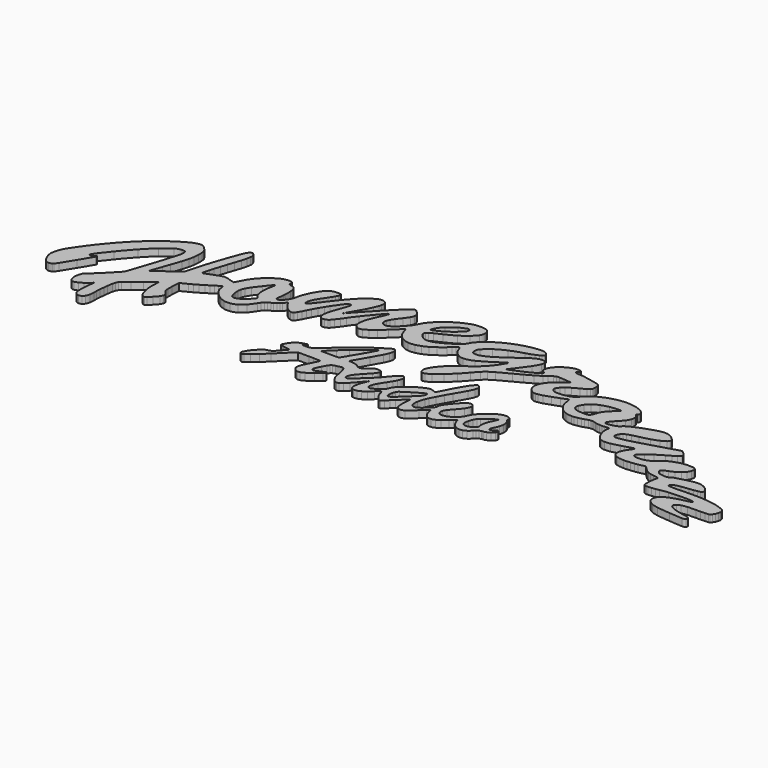
from build123d import *

# Parameters (mm, degrees)
F1_DEPTH = 6


# Not quite as in the source:
# - ends of sketch curves that miss each other by under 0.0002 mm in the source are joined


with BuildPart() as f1:
    # F0 (on Top) → F1 (new body)
    with BuildSketch(Plane.XY):
        with BuildLine():
            ThreePointArc((-4.9511170238, 65.571780151), (-7.0697776136, 65.1364511574), (-9.1387680237, 64.5059650664))
            ThreePointArc((-9.1387680237, 64.5059650664), (-13.4587918929, 62.7453261986), (-17.6046359984, 60.6065339971))
            ThreePointArc((-17.6046359984, 60.6065339971), (-21.63099808, 58.065822324), (-25.429998859, 55.1962578288))
            ThreePointArc((-25.429998859, 55.1962578288), (-28.7595936165, 52.1981272672), (-31.811829985, 48.9180599873))
            ThreePointArc((-31.811829985, 48.9180599873), (-34.1001388015, 45.8196485241), (-35.9394013902, 42.4353281783))
            ThreePointArc((-35.9394013902, 42.4353281783), (-36.9452117725, 40.5244074024), (-38.1577530072, 38.7375060055))
            ThreePointArc((-38.1577530072, 38.7375060055), (-39.8839402891, 36.6009827451), (-41.725036226, 34.5626452157))
            ThreePointArc((-41.725036226, 34.5626452157), (-43.6817525284, 32.622434623), (-45.7422302175, 30.792793259))
            ThreePointArc((-45.7422302175, 30.792793259), (-47.4929934874, 29.4770928074), (-49.3757113331, 28.3583376366))
            ThreePointArc((-49.3757113331, 28.3583376366), (-50.4066044706, 27.9560636842), (-51.5004270333, 27.7883817905))
            ThreePointArc((-51.5004270333, 27.7883817905), (-52.5646752459, 27.8737864998), (-53.5766120763, 28.2142308407))
            ThreePointArc((-53.5766120763, 28.2142308407), (-54.4117925887, 28.7629435386), (-55.0710798719, 29.513911085))
            ThreePointArc((-55.0710798719, 29.513911085), (-55.484034314, 30.3922869798), (-55.625711, 31.352497))
            ThreePointArc((-55.625711, 31.352497), (-55.5397910419, 32.434553781), (-55.2841851222, 33.4894920401))
            ThreePointArc((-55.2841851222, 33.4894920401), (-54.8245599406, 34.6937850992), (-54.2524438804, 35.8488869335))
            ThreePointArc((-54.2524438804, 35.8488869335), (-53.3323260326, 37.3915509843), (-52.3205140745, 38.8756890542))
            ThreePointArc((-52.3205140745, 38.8756890542), (-50.6665806187, 41.1093286776), (-48.9739737402, 43.3138067969))
            ThreePointArc((-48.9739737402, 43.3138067969), (-47.4104463855, 45.4157749255), (-45.9494202828, 47.5902381803))
            ThreePointArc((-45.9494202828, 47.5902381803), (-45.2578563293, 48.975149708), (-44.868750983, 50.4734279974))
            ThreePointArc((-44.868750983, 50.4734279974), (-44.8722949613, 51.7410143915), (-45.2559912214, 52.9491388903))
            ThreePointArc((-45.2559912214, 52.9491388903), (-46.0886913861, 54.3645943128), (-47.115589485, 55.6461495506))
            ThreePointArc((-47.115589485, 55.6461495506), (-47.7938937333, 56.3450749242), (-48.5036457103, 57.0120423229))
            ThreePointArc((-48.5036457103, 57.0120423229), (-48.9763162795, 57.3610297638), (-49.5065520565, 57.6141298452))
            ThreePointArc((-49.5065520565, 57.6141298452), (-49.9756099236, 57.7149110212), (-50.4543549056, 57.6836805426))
            ThreePointArc((-50.4543549056, 57.6836805426), (-51.0319206473, 57.520410968), (-51.5800950662, 57.2759851237))
            ThreePointArc((-51.5800950662, 57.2759851237), (-53.0138888269, 56.3836364149), (-54.3192452851, 55.3121443044))
            ThreePointArc((-54.3192452851, 55.3121443044), (-57.2947852204, 52.4900205752), (-60.2344631435, 49.6305601457))
            ThreePointArc((-60.2344631435, 49.6305601457), (-63.8363228932, 46.0283436054), (-67.3832500963, 42.372025092))
            ThreePointArc((-67.3832500963, 42.372025092), (-71.4430869129, 38.0814635882), (-75.4609509191, 33.7515719257))
            Line((-75.4609509191, 33.7515719257), (-84.650094, 23.751572))
            Line((-84.650094, 23.751572), (-78.555182, 34.408858))
            ThreePointArc((-78.555182, 34.408858), (-77.3007123461, 36.6568765969), (-76.0937775102, 38.9307697466))
            ThreePointArc((-76.0937775102, 38.9307697466), (-75.0312576199, 41.0536434584), (-74.0259971207, 43.2042230545))
            ThreePointArc((-74.0259971207, 43.2042230545), (-73.2377371962, 45.0169294566), (-72.499347882, 46.8505159544))
            ThreePointArc((-72.499347882, 46.8505159544), (-72.1407182895, 47.9693101539), (-71.9161939877, 49.1225249983))
            ThreePointArc((-71.9161939877, 49.1225249983), (-71.7804540425, 50.3019370282), (-71.6890148952, 51.4856079939))
            ThreePointArc((-71.6890148952, 51.4856079939), (-71.7204499535, 52.1103124731), (-71.8858049131, 52.7135550343))
            ThreePointArc((-71.8858049131, 52.7135550343), (-72.157205783, 53.1839337674), (-72.553383104, 53.5553608499))
            ThreePointArc((-72.553383104, 53.5553608499), (-73.2531646524, 53.9954456606), (-73.9893838808, 54.3714112615))
            ThreePointArc((-73.9893838808, 54.3714112615), (-76.5742012472, 54.923300415), (-79.1512520404, 54.3362130856))
            ThreePointArc((-79.1512520404, 54.3362130856), (-82.7466843322, 52.3512204208), (-86.0628074254, 49.928276511))
            ThreePointArc((-86.0628074254, 49.928276511), (-90.4487892511, 45.946464258), (-94.4778620514, 41.6038570437))
            ThreePointArc((-94.4778620514, 41.6038570437), (-99.5803077189, 35.3904681908), (-104.4612051422, 29.0015721048))
            ThreePointArc((-104.4612051422, 29.0015721048), (-105.8616448028, 27.1244166524), (-107.2851189404, 25.2646679538))
            ThreePointArc((-107.2851189404, 25.2646679538), (-108.5395409277, 23.6780407766), (-109.8240043238, 22.1156342715))
            ThreePointArc((-109.8240043238, 22.1156342715), (-110.9236988786, 20.8153347781), (-112.034767888, 19.5247409027))
            ThreePointArc((-112.034767888, 19.5247409027), (-112.3046441643, 19.3230869079), (-112.63386, 19.251572))
            ThreePointArc((-112.63386, 19.251572), (-113.1534578311, 19.4339020312), (-113.4451909434, 19.9009330127))
            ThreePointArc((-113.4451909434, 19.9009330127), (-113.5780961946, 20.8379847705), (-113.560062248, 21.7842429253))
            ThreePointArc((-113.560062248, 21.7842429253), (-113.3577785428, 23.0722381086), (-113.0109219276, 24.3290359755))
            ThreePointArc((-113.0109219276, 24.3290359755), (-112.5007624335, 25.639170388), (-111.8741569222, 26.8977729568))
            ThreePointArc((-111.8741569222, 26.8977729568), (-111.4227784189, 27.6887071372), (-110.9535549252, 28.4691869539))
            ThreePointArc((-110.9535549252, 28.4691869539), (-110.2601497092, 29.583575877), (-109.5579669758, 30.6924549846))
            ThreePointArc((-109.5579669758, 30.6924549846), (-108.774781418, 31.9079921418), (-107.9820923281, 33.1173532169))
            ThreePointArc((-107.9820923281, 33.1173532169), (-107.2184993547, 34.2610649561), (-106.4445191937, 35.3977731332))
            ThreePointArc((-106.4445191937, 35.3977731332), (-105.7148022522, 36.487239477), (-105.0118393347, 37.5941572069))
            ThreePointArc((-105.0118393347, 37.5941572069), (-104.3663786738, 38.6715368655), (-103.751028954, 39.7663935189))
            ThreePointArc((-103.751028954, 39.7663935189), (-103.2553920754, 40.706737649), (-102.7845629329, 41.6597449679))
            ThreePointArc((-102.7845629329, 41.6597449679), (-102.5752078541, 42.1934083931), (-102.4445183252, 42.7515718924))
            ThreePointArc((-102.4445183252, 42.7515718924), (-102.4077864665, 43.2814269159), (-102.4653039606, 43.8094300079))
            ThreePointArc((-102.4653039606, 43.8094300079), (-102.6225119539, 44.1538255315), (-102.9166821282, 44.3921247346))
            ThreePointArc((-102.9166821282, 44.3921247346), (-103.4336994969, 44.5779323749), (-103.9780899869, 44.6518954353))
            ThreePointArc((-103.9780899869, 44.6518954353), (-105.1900611805, 44.672961912), (-106.4021770036, 44.6633081759))
            ThreePointArc((-106.4021770036, 44.6633081759), (-107.5224980274, 44.6034536689), (-108.636502092, 44.470424602))
            ThreePointArc((-108.636502092, 44.470424602), (-109.5365151488, 44.2782129063), (-110.4077529115, 43.9817107827))
            ThreePointArc((-110.4077529115, 43.9817107827), (-111.2301884152, 43.5879986198), (-111.9999349885, 43.099224984))
            ThreePointArc((-111.9999349885, 43.099224984), (-112.8651566082, 42.4276814487), (-113.6817990251, 41.6978360262))
            ThreePointArc((-113.6817990251, 41.6978360262), (-115.242220676, 40.0158598094), (-116.5941946224, 38.1621807573))
            ThreePointArc((-116.5941946224, 38.1621807573), (-118.1458386997, 35.5989311319), (-119.5572610139, 32.955877007))
            ThreePointArc((-119.5572610139, 32.955877007), (-120.8411833252, 30.2044843673), (-121.9750042553, 27.3879140949))
            ThreePointArc((-121.9750042553, 27.3879140949), (-122.7037564143, 25.0652486809), (-123.1887528616, 22.6797439792))
            ThreePointArc((-123.1887528616, 22.6797439792), (-123.5931985562, 20.8617023035), (-124.2475459185, 19.1179474202))
            ThreePointArc((-124.2475459185, 19.1179474202), (-125.187143212, 17.3311891664), (-126.31751175, 15.6585818102))
            ThreePointArc((-126.31751175, 15.6585818102), (-127.4884363203, 14.291398953), (-128.8117564177, 13.0711215101))
            ThreePointArc((-128.8117564177, 13.0711215101), (-129.8880841133, 12.4626072966), (-131.106376, 12.251572))
            ThreePointArc((-131.106376, 12.251572), (-131.5035761773, 12.2898275292), (-131.8861740138, 12.4031869658))
            ThreePointArc((-131.8861740138, 12.4031869658), (-132.144822049, 12.5736153993), (-132.3174273034, 12.8308158744))
            ThreePointArc((-132.3174273034, 12.8308158744), (-132.4264352389, 13.2208728402), (-132.439613499, 13.6256609561))
            ThreePointArc((-132.439613499, 13.6256609561), (-132.3605229139, 14.3162073943), (-132.2448293927, 15.0015720771))
            ThreePointArc((-132.2448293927, 15.0015720771), (-132.1284334207, 15.6348798209), (-132.0273483382, 16.2708110496))
            ThreePointArc((-132.0273483382, 16.2708110496), (-131.9188539063, 17.0472148151), (-131.8208236212, 17.825009074))
            ThreePointArc((-131.8208236212, 17.825009074), (-131.7321883317, 18.6135781314), (-131.6541477484, 19.4032660689))
            ThreePointArc((-131.6541477484, 19.4032660689), (-131.5994838006, 20.0769064176), (-131.5594114762, 20.7515720231))
            ThreePointArc((-131.5594114762, 20.7515720231), (-131.4831168027, 23.7211340906), (-131.542374105, 26.6910849955))
            ThreePointArc((-131.542374105, 26.6910849955), (-131.7763347754, 28.59032288), (-132.3091669403, 30.4282380226))
            ThreePointArc((-132.3091669403, 30.4282380226), (-132.9589122939, 31.6119440072), (-133.9105280557, 32.5699399266))
            ThreePointArc((-133.9105280557, 32.5699399266), (-135.0825365807, 33.2183491414), (-136.3900879656, 33.5087764571))
            ThreePointArc((-136.3900879656, 33.5087764571), (-136.8150894027, 33.5600344621), (-137.2337919222, 33.6491512991))
            ThreePointArc((-137.2337919222, 33.6491512991), (-137.5905710527, 33.7675996957), (-137.9286588805, 33.9319712094))
            ThreePointArc((-137.9286588805, 33.9319712094), (-138.1693747176, 34.0988136264), (-138.3773383288, 34.3050457219))
            ThreePointArc((-138.3773383288, 34.3050457219), (-138.4818460344, 34.4966822002), (-138.5022818958, 34.7140039886))
            ThreePointArc((-138.5022818958, 34.7140039886), (-138.4463059214, 35.616876144), (-138.4754566024, 36.5210120316))
            ThreePointArc((-138.4754566024, 36.5210120316), (-138.6172086538, 37.0746113239), (-138.9367579654, 37.5483770332))
            ThreePointArc((-138.9367579654, 37.5483770332), (-139.4065172496, 37.9009556418), (-139.9641479997, 38.0854370021))
            ThreePointArc((-139.9641479997, 38.0854370021), (-140.9169710024, 38.1967496844), (-141.8757109999, 38.229609982))
            ThreePointArc((-141.8757109999, 38.229609982), (-145.0843366816, 37.8540699973), (-148.1341987043, 36.7888703811))
            ThreePointArc((-148.1341987043, 36.7888703811), (-151.7183069584, 34.8266161198), (-155.0646739726, 32.4818129652))
            ThreePointArc((-155.0646739726, 32.4818129652), (-158.4221910339, 29.5488712763), (-161.459265495, 26.2852465766))
            ThreePointArc((-161.459265495, 26.2852465766), (-164.0189565886, 22.8454360914), (-166.1629380524, 19.1322625239))
            ThreePointArc((-166.1629380524, 19.1322625239), (-166.6894764177, 18.0887025546), (-167.2195686511, 17.0469433327))
            ThreePointArc((-167.2195686511, 17.0469433327), (-167.6853998756, 16.1410727899), (-168.1558799679, 15.2376079832))
            ThreePointArc((-168.1558799679, 15.2376079832), (-168.5623917287, 14.4637563471), (-168.9704654023, 13.6907272129))
            ThreePointArc((-168.9704654023, 13.6907272129), (-169.0530598807, 13.5548467324), (-169.1511917248, 13.4297247564))
            ThreePointArc((-169.1511917248, 13.4297247564), (-169.2667156869, 13.3542515119), (-169.4045768304, 13.3482337446))
            ThreePointArc((-169.4045768304, 13.3482337446), (-170.0533282283, 13.5001582885), (-170.700173145, 13.6600054282))
            ThreePointArc((-170.700173145, 13.6600054282), (-171.4751955351, 13.8665549365), (-172.2450041131, 14.09175963))
            ThreePointArc((-172.2450041131, 14.09175963), (-173.1368367815, 14.3718777929), (-174.0242768428, 14.6656154631))
            ThreePointArc((-174.0242768428, 14.6656154631), (-175.4643651074, 15.1193545721), (-176.9230691461, 15.5091184004))
            ThreePointArc((-176.9230691461, 15.5091184004), (-177.879796806, 15.6646361021), (-178.8490679575, 15.6698334147))
            ThreePointArc((-178.8490679575, 15.6698334147), (-179.917609449, 15.525964763), (-180.9605319025, 15.2524837035))
            ThreePointArc((-180.9605319025, 15.2524837035), (-182.9218489892, 14.5850809114), (-184.8690961058, 13.8776772821))
            ThreePointArc((-184.8690961058, 13.8776772821), (-186.1301093264, 13.4032456214), (-187.3900222003, 12.9258995268))
            ThreePointArc((-187.3900222003, 12.9258995268), (-188.5909717162, 12.4674719497), (-189.7906969233, 12.0058498015))
            ThreePointArc((-189.7906969233, 12.0058498015), (-190.8065917372, 11.6120137603), (-191.8215439448, 11.2157548592))
            ThreePointArc((-191.8215439448, 11.2157548592), (-192.3311807101, 11.0115197163), (-192.8375970587, 10.7994251372))
            ThreePointArc((-192.8375970587, 10.7994251372), (-193.2345411499, 10.7043849311), (-193.6405119555, 10.746633159))
            ThreePointArc((-193.6405119555, 10.746633159), (-193.8998303005, 10.9263441873), (-193.9927103451, 11.2278660118))
            ThreePointArc((-193.9927103451, 11.2278660118), (-193.9248798341, 11.976451658), (-193.7735204445, 12.7127068528))
            ThreePointArc((-193.7735204445, 12.7127068528), (-193.2088610552, 14.8130636704), (-192.6287625875, 16.9092088842))
            ThreePointArc((-192.6287625875, 16.9092088842), (-192.1330628133, 18.6336442621), (-191.6158741187, 20.3517570365))
            ThreePointArc((-191.6158741187, 20.3517570365), (-190.852936323, 22.8108796972), (-190.079205796, 25.2666279352))
            ThreePointArc((-190.079205796, 25.2666279352), (-189.2166688968, 27.963026096), (-188.3423838773, 30.6556379599))
            ThreePointArc((-188.3423838773, 30.6556379599), (-187.5009988934, 33.2057696411), (-186.646603933, 35.7515719773))
            ThreePointArc((-186.646603933, 35.7515719773), (-185.7286657679, 38.5298342226), (-184.8510668169, 41.3211012504))
            ThreePointArc((-184.8510668169, 41.3211012504), (-184.2492585412, 43.412575706), (-183.719766618, 45.5235179111))
            ThreePointArc((-183.719766618, 45.5235179111), (-183.3917477448, 47.0845608005), (-183.1309486261, 48.65823009))
            ThreePointArc((-183.1309486261, 48.65823009), (-183.0797069117, 49.6167685256), (-183.1997335721, 50.5691420933))
            ThreePointArc((-183.1997335721, 50.5691420933), (-183.5275906799, 51.6604926451), (-184.0191346557, 52.6885591985))
            ThreePointArc((-184.0191346557, 52.6885591985), (-184.5817370666, 53.3883554405), (-185.3300801196, 53.8845597402))
            ThreePointArc((-185.3300801196, 53.8845597402), (-186.0687989447, 54.0551331195), (-186.8144200733, 53.91783718))
            ThreePointArc((-186.8144200733, 53.91783718), (-187.5666997477, 53.4822910756), (-188.1715627943, 52.8579788496))
            ThreePointArc((-188.1715627943, 52.8579788496), (-189.292279701, 51.088050859), (-190.166872948, 49.1844389802))
            ThreePointArc((-190.166872948, 49.1844389802), (-192.1644808364, 43.8570145716), (-194.1083309472, 38.5097409811))
            ThreePointArc((-194.1083309472, 38.5097409811), (-196.119501099, 32.7509577038), (-198.0424241004, 26.9621100325))
            ThreePointArc((-198.0424241004, 26.9621100325), (-199.6253806243, 21.8742773835), (-201.0915596631, 16.7515719077))
            Line((-201.0915596631, 16.7515719077), (-204.378103, 4.751572))
            Line((-204.378103, 4.751572), (-213.751907, -1.995131))
            ThreePointArc((-213.751907, -1.995131), (-215.5550852535, -3.290318478), (-217.3607525548, -4.5820336236))
            ThreePointArc((-217.3607525548, -4.5820336236), (-218.8952629556, -5.6739079896), (-220.4331939136, -6.7609591227))
            ThreePointArc((-220.4331939136, -6.7609591227), (-221.8072474289, -7.7285889629), (-223.181637755, -8.6957403483))
            ThreePointArc((-223.181637755, -8.6957403483), (-223.2538550689, -8.7318562748), (-223.3335010022, -8.7451308588))
            ThreePointArc((-223.3335010022, -8.7451308588), (-223.3823549282, -8.7207506345), (-223.3905379646, -8.666768012))
            ThreePointArc((-223.3905379646, -8.666768012), (-222.6159141736, -6.3937202689), (-221.8406315981, -4.1208971371))
            ThreePointArc((-221.8406315981, -4.1208971371), (-220.9675128796, -1.5777350907), (-220.0850711725, 0.9622070603))
            ThreePointArc((-220.0850711725, 0.9622070603), (-219.0256344033, 3.9830499738), (-217.9596029105, 7.0015719683))
            ThreePointArc((-217.9596029105, 7.0015719683), (-216.5059728006, 11.1734285956), (-215.0966535332, 15.3604618456))
            ThreePointArc((-215.0966535332, 15.3604618456), (-214.2319595618, 18.1377484845), (-213.4652390673, 20.9436630171))
            ThreePointArc((-213.4652390673, 20.9436630171), (-212.9729001114, 23.110825417), (-212.5930110673, 25.3005000099))
            ThreePointArc((-212.5930110673, 25.3005000099), (-212.356776245, 27.3600755281), (-212.2518131981, 29.4304960037))
            ThreePointArc((-212.2518131981, 29.4304960037), (-212.2381577403, 31.4222392254), (-212.2723934762, 33.4137350153))
            ThreePointArc((-212.2723934762, 33.4137350153), (-212.3735500804, 34.4986889665), (-212.6118498101, 35.5619720555))
            ThreePointArc((-212.6118498101, 35.5619720555), (-212.9524236538, 36.4384580493), (-213.4386036079, 37.243347557))
            ThreePointArc((-213.4386036079, 37.243347557), (-214.2492731239, 38.2830731408), (-215.12571142, 39.267994601))
            ThreePointArc((-215.12571142, 39.267994601), (-215.9939012426, 40.1380158481), (-216.9039753465, 40.9641245988))
            ThreePointArc((-216.9039753465, 40.9641245988), (-217.5493607352, 41.4323621098), (-218.2644769727, 41.7850340698))
            ThreePointArc((-218.2644769727, 41.7850340698), (-218.9949553827, 41.9955973581), (-219.7517419998, 42.0677750869))
            ThreePointArc((-219.7517419998, 42.0677750869), (-220.8364832107, 42.0342304444), (-221.9166040781, 41.9287425944))
            ThreePointArc((-221.9166040781, 41.9287425944), (-224.1198014914, 41.4607938495), (-226.2223942006, 40.6532304201))
            ThreePointArc((-226.2223942006, 40.6532304201), (-229.4190145782, 39.0431625785), (-232.5446242668, 37.2992404553))
            ThreePointArc((-232.5446242668, 37.2992404553), (-236.1730231401, 35.0730659164), (-239.7084241045, 32.7019751491))
            ThreePointArc((-239.7084241045, 32.7019751491), (-243.3879933087, 30.0325920145), (-246.9768469635, 27.2424369546))
            ThreePointArc((-246.9768469635, 27.2424369546), (-254.3022396327, 20.9284959863), (-261.1827458995, 14.1324779049))
            ThreePointArc((-261.1827458995, 14.1324779049), (-268.4189088612, 6.1006047665), (-275.2559274472, -2.2736544293))
            ThreePointArc((-275.2559274472, -2.2736544293), (-281.0947416556, -10.1482200046), (-286.5761189353, -18.2756450416))
            ThreePointArc((-286.5761189353, -18.2756450416), (-289.0060690099, -23.1895095536), (-290.2861420315, -28.5198129961))
            ThreePointArc((-290.2861420315, -28.5198129961), (-290.3584540634, -30.5440165288), (-290.0744244711, -32.5494981098))
            ThreePointArc((-290.0744244711, -32.5494981098), (-289.419898514, -34.7378523706), (-288.5008443852, -36.8289376832))
            ThreePointArc((-288.5008443852, -36.8289376832), (-287.4302019252, -38.6084219346), (-286.1352923664, -40.2320133339))
            ThreePointArc((-286.1352923664, -40.2320133339), (-284.9732253785, -41.1205655685), (-283.5735349761, -41.5457607951))
            ThreePointArc((-283.5735349761, -41.5457607951), (-283.0057295858, -41.5765975015), (-282.4384480995, -41.5372842441))
            ThreePointArc((-282.4384480995, -41.5372842441), (-281.8518659064, -41.4278961786), (-281.2803048145, -41.2565415165))
            ThreePointArc((-281.2803048145, -41.2565415165), (-280.7387162502, -41.0282334977), (-280.2250178572, -40.742652227))
            ThreePointArc((-280.2250178572, -40.742652227), (-279.785716108, -40.4223434408), (-279.3942056961, -40.045112275))
            ThreePointArc((-279.3942056961, -40.045112275), (-278.3017210632, -38.7219886213), (-277.3335860958, -37.3053399407))
            ThreePointArc((-277.3335860958, -37.3053399407), (-274.0713620901, -32.0120078135), (-270.8285440846, -26.7067649485))
            ThreePointArc((-270.8285440846, -26.7067649485), (-267.4022817797, -21.0691685786), (-263.9841299807, -15.4266510117))
            ThreePointArc((-263.9841299807, -15.4266510117), (-263.7169936876, -14.8085727003), (-263.625711, -14.141452))
            ThreePointArc((-263.625711, -14.141452), (-263.6768493039, -14.0353912761), (-263.7916799446, -14.0093542405))
            ThreePointArc((-263.7916799446, -14.0093542405), (-264.0925828483, -14.0919614365), (-264.3855728577, -14.1993083435))
            ThreePointArc((-264.3855728577, -14.1993083435), (-264.8089046113, -14.3902573786), (-265.2196319097, -14.606993159))
            ThreePointArc((-265.2196319097, -14.606993159), (-265.7208727276, -14.9022656665), (-266.2124748196, -15.2133212753))
            ThreePointArc((-266.2124748196, -15.2133212753), (-267.2493602621, -15.7001718391), (-268.3807909994, -15.8791110394))
            ThreePointArc((-268.3807909994, -15.8791110394), (-268.9300651786, -15.5781284808), (-268.9522175945, -14.9521876892))
            ThreePointArc((-268.9522175945, -14.9521876892), (-267.6489081144, -12.7058346116), (-266.1530929915, -10.5828050065))
            ThreePointArc((-266.1530929915, -10.5828050065), (-262.6909268156, -6.1525408745), (-259.1799489048, -1.760859077))
            ThreePointArc((-259.1799489048, -1.760859077), (-253.9188662509, 4.5451203483), (-248.4665300198, 10.6864880181))
            ThreePointArc((-248.4665300198, 10.6864880181), (-243.7536534826, 15.5612993103), (-238.783507738, 20.1735267019))
            ThreePointArc((-238.783507738, 20.1735267019), (-234.7746588362, 23.4839419277), (-230.5702910252, 26.542211037))
            ThreePointArc((-230.5702910252, 26.542211037), (-227.9272354902, 27.8145291138), (-225.026627, 28.251572))
            ThreePointArc((-225.026627, 28.251572), (-224.013660159, 28.2283489012), (-223.0028219977, 28.1587260249))
            ThreePointArc((-223.0028219977, 28.1587260249), (-222.5371537076, 28.0348028734), (-222.1386008465, 27.7639531598))
            ThreePointArc((-222.1386008465, 27.7639531598), (-221.8607949736, 27.3818532044), (-221.7325390707, 26.927180993))
            ThreePointArc((-221.7325390707, 26.927180993), (-221.6629721018, 25.9655319167), (-221.6432286894, 25.0015719983))
            ThreePointArc((-221.6432286894, 25.0015719983), (-221.7192642358, 23.9205013901), (-221.9344336066, 22.8583351644))
            ThreePointArc((-221.9344336066, 22.8583351644), (-222.7997965658, 19.714414668), (-223.6896498706, 16.5773379628))
            ThreePointArc((-223.6896498706, 16.5773379628), (-224.7889667092, 12.8401804449), (-225.9315069463, 9.1160099832))
            ThreePointArc((-225.9315069463, 9.1160099832), (-227.2408811844, 4.9959548158), (-228.5851701937, 0.8871590643))
            Line((-228.5851701937, 0.8871590643), (-235.509593, -19.977255))
            Line((-235.509593, -19.977255), (-242.817652, -27.611263))
            ThreePointArc((-242.817652, -27.611263), (-244.305507197, -29.1450541961), (-245.8135081075, -30.6590428915))
            ThreePointArc((-245.8135081075, -30.6590428915), (-247.2820654719, -32.0925139003), (-248.7718511673, -33.5039098208))
            ThreePointArc((-248.7718511673, -33.5039098208), (-250.0546535741, -34.6847435552), (-251.3536078991, -35.8477861143))
            ThreePointArc((-251.3536078991, -35.8477861143), (-252.0672055522, -36.4289026641), (-252.8248860717, -36.9512418866))
            ThreePointArc((-252.8248860717, -36.9512418866), (-254.4791136005, -38.3635131847), (-255.6676625091, -40.1851417634))
            ThreePointArc((-255.6676625091, -40.1851417634), (-256.5527404687, -42.6167104734), (-257.0085762056, -45.1638859812))
            ThreePointArc((-257.0085762056, -45.1638859812), (-256.998071234, -47.5338331138), (-256.5377825452, -49.8586758638))
            ThreePointArc((-256.5377825452, -49.8586758638), (-255.6734636704, -51.3706020377), (-254.2309759572, -52.3464078884))
            ThreePointArc((-254.2309759572, -52.3464078884), (-253.3841278119, -52.5152507302), (-252.5293549087, -52.3926822831))
            ThreePointArc((-252.5293549087, -52.3926822831), (-251.0549013098, -51.8628410638), (-249.6185347101, -51.2370646098))
            ThreePointArc((-249.6185347101, -51.2370646098), (-248.0222375185, -50.4100511201), (-246.4861789646, -49.475899054))
            ThreePointArc((-246.4861789646, -49.475899054), (-245.0955900372, -48.4823742428), (-243.7883768304, -47.3814551858))
            Line((-243.7883768304, -47.3814551858), (-241.451044, -45.248428))
            Line((-241.451044, -45.248428), (-242.154337, -53.347497))
            ThreePointArc((-242.154337, -53.347497), (-242.3559360688, -56.363955393), (-242.4374462919, -59.3860439979))
            ThreePointArc((-242.4374462919, -59.3860439979), (-242.3031200096, -61.2272666607), (-241.8775132753, -63.0236527658))
            ThreePointArc((-241.8775132753, -63.0236527658), (-241.320749436, -64.1219191583), (-240.4525969544, -64.9951239377))
            ThreePointArc((-240.4525969544, -64.9951239377), (-239.35989135, -65.5553270156), (-238.147231, -65.748428))
            ThreePointArc((-238.147231, -65.748428), (-236.9457742434, -65.5751803201), (-235.8422098898, -65.0695531708))
            ThreePointArc((-235.8422098898, -65.0695531708), (-234.8485893533, -64.2454542568), (-234.0784297898, -63.2094645481))
            ThreePointArc((-234.0784297898, -63.2094645481), (-233.3981698731, -61.7388834828), (-232.9810174377, -60.1732059231))
            ThreePointArc((-232.9810174377, -60.1732059231), (-232.7147058729, -58.1434738905), (-232.625711, -56.098281))
            ThreePointArc((-232.625711, -56.098281), (-232.6076713002, -54.8272630297), (-232.5535670175, -53.557268999))
            ThreePointArc((-232.5535670175, -53.557268999), (-232.4458783162, -51.840112605), (-232.3180621818, -50.1243369854))
            ThreePointArc((-232.3180621818, -50.1243369854), (-232.1594237227, -48.2845864363), (-231.9794740592, -46.4467979939))
            ThreePointArc((-231.9794740592, -46.4467979939), (-231.7914671191, -44.757303655), (-231.578396363, -43.0707869514))
            ThreePointArc((-231.578396363, -43.0707869514), (-231.2686512169, -40.9351759826), (-230.9122626199, -38.8068518892))
            ThreePointArc((-230.9122626199, -38.8068518892), (-230.6236964094, -37.5224727389), (-230.2229836922, -36.2685471135))
            ThreePointArc((-230.2229836922, -36.2685471135), (-229.808292562, -35.3437459364), (-229.2719268224, -34.4837821283))
            ThreePointArc((-229.2719268224, -34.4837821283), (-228.5957730688, -33.6536529246), (-227.8283956133, -32.9070404463))
            ThreePointArc((-227.8283956133, -32.9070404463), (-225.4278830207, -30.8604615536), (-222.9952792535, -28.852132688))
            ThreePointArc((-222.9952792535, -28.852132688), (-219.7096370318, -26.2013473353), (-216.406182285, -23.5727936393))
            ThreePointArc((-216.406182285, -23.5727936393), (-212.8606989158, -20.7742032323), (-209.3122458645, -17.9793791722))
            ThreePointArc((-209.3122458645, -17.9793791722), (-208.9981415144, -17.8077993978), (-208.645188, -17.748428))
            ThreePointArc((-208.645188, -17.748428), (-208.5110216087, -17.8007811242), (-208.4477720616, -17.9301680051))
            ThreePointArc((-208.4477720616, -17.9301680051), (-208.4055240306, -18.5281077542), (-208.3777627228, -19.1268949905))
            ThreePointArc((-208.3777627228, -19.1268949905), (-208.3653081636, -19.8843355696), (-208.3797949276, -20.6417400027))
            ThreePointArc((-208.3797949276, -20.6417400027), (-208.4226084324, -21.541966308), (-208.484521431, -22.4410809657))
            ThreePointArc((-208.484521431, -22.4410809657), (-208.5726876549, -24.8462193576), (-208.4552643274, -27.2501069383))
            ThreePointArc((-208.4552643274, -27.2501069383), (-208.1301276128, -29.8225901908), (-207.6299716207, -32.3668441442))
            ThreePointArc((-207.6299716207, -32.3668441442), (-207.024774084, -34.6173114054), (-206.2662665931, -36.8208388441))
            ThreePointArc((-206.2662665931, -36.8208388441), (-205.5628338854, -38.1613430438), (-204.5670030952, -39.3015581052))
            ThreePointArc((-204.5670030952, -39.3015581052), (-203.9497265641, -39.7870278066), (-203.2714350479, -40.1827950968))
            ThreePointArc((-203.2714350479, -40.1827950968), (-202.76675241, -40.3055291782), (-202.2579653502, -40.2011082219))
            ThreePointArc((-202.2579653502, -40.2011082219), (-201.6001899568, -39.8311916391), (-201.0186698756, -39.3502121257))
            ThreePointArc((-201.0186698756, -39.3502121257), (-199.5563348082, -37.8831486523), (-198.1134384456, -36.3969625312))
            ThreePointArc((-198.1134384456, -36.3969625312), (-196.555892551, -34.6857122923), (-195.0880629128, -32.8969130679))
            ThreePointArc((-195.0880629128, -32.8969130679), (-194.3534488382, -31.7123603015), (-193.8856202679, -30.3993639356))
            ThreePointArc((-193.8856202679, -30.3993639356), (-193.8159841966, -29.3279184016), (-194.1096410832, -28.29515004))
            ThreePointArc((-194.1096410832, -28.29515004), (-194.7865144498, -27.1781558067), (-195.6656627733, -26.2122717495))
            ThreePointArc((-195.6656627733, -26.2122717495), (-196.2419558237, -25.6066516495), (-196.7217649906, -24.9220549944))
            ThreePointArc((-196.7217649906, -24.9220549944), (-197.0696949553, -24.2036367303), (-197.2900622288, -23.436422045))
            ThreePointArc((-197.2900622288, -23.436422045), (-197.4491253935, -22.3471536754), (-197.5007515659, -21.2475439988))
            ThreePointArc((-197.5007515659, -21.2475439988), (-197.4773786684, -19.277000497), (-197.4156633379, -17.3072849861))
            Line((-197.4156633379, -17.3072849861), (-197.125711, -10.248428))
            Line((-197.125711, -10.248428), (-191.125711, -7.170645))
            ThreePointArc((-191.125711, -7.170645), (-189.7401689061, -6.4441560615), (-188.3678686956, -5.6929535444))
            ThreePointArc((-188.3678686956, -5.6929535444), (-186.6827144271, -4.740184238), (-185.0067317761, -3.7713723831))
            ThreePointArc((-185.0067317761, -3.7713723831), (-183.3031895825, -2.7648731442), (-181.6092837566, -1.7422393989))
            ThreePointArc((-181.6092837566, -1.7422393989), (-180.1582705285, -0.8420808116), (-178.7206749593, 0.0793549375))
            ThreePointArc((-178.7206749593, 0.0793549375), (-177.4674414691, 0.8857176287), (-176.2052283088, 1.6779504982))
            ThreePointArc((-176.2052283088, 1.6779504982), (-175.0825783353, 2.361187945), (-173.9489099221, 3.0259828647))
            ThreePointArc((-173.9489099221, 3.0259828647), (-172.9906783391, 3.5715619013), (-172.0274592088, 4.1082863788))
            ThreePointArc((-172.0274592088, 4.1082863788), (-171.7581376766, 4.2151761003), (-171.470675, 4.251572))
            ThreePointArc((-171.470675, 4.251572), (-171.2881651776, 4.2071471051), (-171.1464899775, 4.083812016))
            ThreePointArc((-171.1464899775, 4.083812016), (-170.9924649316, 3.8314672256), (-170.8739189543, 3.5606380164))
            ThreePointArc((-170.8739189543, 3.5606380164), (-170.7607955009, 3.1853774289), (-170.6873072959, 2.8003879594))
            ThreePointArc((-170.6873072959, 2.8003879594), (-170.6411278127, 2.3509730986), (-170.625711, 1.899455))
            ThreePointArc((-170.625711, 1.899455), (-170.3598643864, -0.1373909666), (-169.580138942, -2.0377709668))
            ThreePointArc((-169.580138942, -2.0377709668), (-168.1291529339, -4.2453956542), (-166.4149638124, -6.2555008186))
            ThreePointArc((-166.4149638124, -6.2555008186), (-164.3588929039, -8.1417712659), (-162.0917660621, -9.7682950986))
            ThreePointArc((-162.0917660621, -9.7682950986), (-159.9009948827, -10.8964595415), (-157.5483169473, -11.6293577588))
            ThreePointArc((-157.5483169473, -11.6293577588), (-154.8598546789, -11.9553710512), (-152.1580300443, -11.7702827306))
            ThreePointArc((-152.1580300443, -11.7702827306), (-149.5156261461, -11.0810301877), (-147.0444569369, -9.9188381073))
            ThreePointArc((-147.0444569369, -9.9188381073), (-144.5228866499, -8.1552875855), (-142.3079960052, -6.0192429954))
            ThreePointArc((-142.3079960052, -6.0192429954), (-140.0295557428, -3.1853302366), (-138.0324196602, -0.14661361))
            ThreePointArc((-138.0324196602, -0.14661361), (-137.4133420768, 0.8208536793), (-136.7268941072, 1.741744086))
            ThreePointArc((-136.7268941072, 1.741744086), (-135.9920799943, 2.5888340165), (-135.1945717312, 3.3771827064))
            ThreePointArc((-135.1945717312, 3.3771827064), (-134.3540952829, 4.0883184496), (-133.4606633427, 4.7316645175))
            ThreePointArc((-133.4606633427, 4.7316645175), (-132.5289836068, 5.2960585105), (-131.5548469173, 5.7835268165))
            ThreePointArc((-131.5548469173, 5.7835268165), (-130.6787872109, 6.2103400765), (-129.8296288523, 6.688440755))
            ThreePointArc((-129.8296288523, 6.688440755), (-128.9008407666, 7.2750211512), (-127.9972342735, 7.8996963785))
            ThreePointArc((-127.9972342735, 7.8996963785), (-127.151147021, 8.5385046773), (-126.332688882, 9.2123488627))
            ThreePointArc((-126.332688882, 9.2123488627), (-125.7106506121, 9.7920712841), (-125.1373859116, 10.4200659256))
            Line((-125.1373859116, 10.4200659256), (-122.774433, 13.228277))
            Line((-122.774433, 13.228277), (-120.603529, 9.71568))
            ThreePointArc((-120.603529, 9.71568), (-119.6462227361, 8.3483830494), (-118.5389751587, 7.0994078422))
            ThreePointArc((-118.5389751587, 7.0994078422), (-117.2888730994, 5.9757844184), (-115.9209016064, 4.9990866223))
            ThreePointArc((-115.9209016064, 4.9990866223), (-114.6516287001, 4.3036041228), (-113.3053099517, 3.7724021491))
            ThreePointArc((-113.3053099517, 3.7724021491), (-112.2941059047, 3.626589983), (-111.2921109786, 3.8260919442))
            ThreePointArc((-111.2921109786, 3.8260919442), (-110.8750608093, 4.0614370819), (-110.5443483628, 4.4077712562))
            ThreePointArc((-110.5443483628, 4.4077712562), (-109.8620270698, 5.4013929304), (-109.2062358055, 6.4127208775))
            ThreePointArc((-109.2062358055, 6.4127208775), (-108.4441021944, 7.6678427373), (-107.7233896821, 8.9471988277))
            ThreePointArc((-107.7233896821, 8.9471988277), (-106.9652193294, 10.3870646343), (-106.2418804924, 11.8447397557))
            ThreePointArc((-106.2418804924, 11.8447397557), (-105.3988081655, 13.5438601022), (-104.5152594054, 15.2222886779))
            ThreePointArc((-104.5152594054, 15.2222886779), (-103.4065381129, 17.2358928403), (-102.2706224642, 19.234282268))
            ThreePointArc((-102.2706224642, 19.234282268), (-101.0970065317, 21.2354248821), (-99.8964321028, 23.2205110631))
            ThreePointArc((-99.8964321028, 23.2205110631), (-98.8484149573, 24.8856749695), (-97.763893646, 26.5272974371))
            ThreePointArc((-97.763893646, 26.5272974371), (-94.6566347467, 31.0244409905), (-91.4621664613, 35.460061604))
            ThreePointArc((-91.4621664613, 35.460061604), (-90.2949492589, 36.4631466611), (-88.8060739985, 36.852795947))
            ThreePointArc((-88.8060739985, 36.852795947), (-87.8533696988, 36.4009648708), (-87.6601660831, 35.3643990246))
            ThreePointArc((-87.6601660831, 35.3643990246), (-89.0161128478, 31.0289496978), (-90.506255226, 26.7377740825))
            ThreePointArc((-90.506255226, 26.7377740825), (-91.5566635373, 23.7747284478), (-92.552945678, 20.7930478957))
            ThreePointArc((-92.552945678, 20.7930478957), (-93.0989503517, 18.8905798864), (-93.5148855798, 16.9555079245))
            ThreePointArc((-93.5148855798, 16.9555079245), (-93.6931508063, 15.5236029058), (-93.7160708495, 14.0808260057))
            ThreePointArc((-93.7160708495, 14.0808260057), (-93.5725672918, 12.7743703858), (-93.2448424245, 11.5015718577))
            ThreePointArc((-93.2448424245, 11.5015718577), (-92.8688306374, 10.7298174158), (-92.3069818542, 10.0807291638))
            ThreePointArc((-92.3069818542, 10.0807291638), (-91.6044944627, 9.6086861301), (-90.8012269643, 9.3420881907))
            ThreePointArc((-90.8012269643, 9.3420881907), (-89.8149929119, 9.2656664447), (-88.8351659765, 9.4014499061))
            ThreePointArc((-88.8351659765, 9.4014499061), (-87.6954329296, 9.762475542), (-86.6086488664, 10.2607037503))
            ThreePointArc((-86.6086488664, 10.2607037503), (-86.0520165053, 10.6277267948), (-85.5714997795, 11.0899488093))
            ThreePointArc((-85.5714997795, 11.0899488093), (-84.5189185825, 12.328309091), (-83.4882587151, 13.5849727705))
            ThreePointArc((-83.4882587151, 13.5849727705), (-82.27895191, 15.1203125719), (-81.103595145, 16.6817951067))
            ThreePointArc((-81.103595145, 16.6817951067), (-79.8540634127, 18.4106229615), (-78.6338799327, 20.1602879539))
            ThreePointArc((-78.6338799327, 20.1602879539), (-76.18072776, 23.6192545285), (-73.6157543778, 26.9961342968))
            ThreePointArc((-73.6157543778, 26.9961342968), (-70.5429469578, 30.8230389184), (-67.3898369777, 34.5840549809))
            ThreePointArc((-67.3898369777, 34.5840549809), (-64.2252831323, 38.254620572), (-61.0371787971, 41.9047498217))
            ThreePointArc((-61.0371787971, 41.9047498217), (-60.5157212791, 42.150804817), (-59.9795423597, 41.9387356403))
            ThreePointArc((-59.9795423597, 41.9387356403), (-59.8927912386, 41.7787774619), (-59.907330011, 41.5973910042))
            ThreePointArc((-59.907330011, 41.5973910042), (-60.3358268136, 40.4993897557), (-60.7722880467, 39.4045300188))
            ThreePointArc((-60.7722880467, 39.4045300188), (-61.3053848402, 38.1160057117), (-61.8623865856, 36.8376332617))
            ThreePointArc((-61.8623865856, 36.8376332617), (-62.5385837442, 35.3475435226), (-63.2319794762, 33.8653787512))
            ThreePointArc((-63.2319794762, 33.8653787512), (-64.6641740745, 30.6571656009), (-65.9440846803, 27.3852178835))
            ThreePointArc((-65.9440846803, 27.3852178835), (-66.7526007318, 24.7738318236), (-67.3010433496, 22.0957268998))
            ThreePointArc((-67.3010433496, 22.0957268998), (-67.4746818563, 20.0533825545), (-67.3696095844, 18.0063650498))
            ThreePointArc((-67.3696095844, 18.0063650498), (-66.9523696147, 16.5184150524), (-66.1035381114, 15.2270708992))
            ThreePointArc((-66.1035381114, 15.2270708992), (-65.7218577383, 14.834799806), (-65.312837978, 14.4711250267))
            ThreePointArc((-65.312837978, 14.4711250267), (-64.8761470461, 14.13559415), (-64.416761733, 13.8318754367))
            ThreePointArc((-64.416761733, 13.8318754367), (-63.9921915311, 13.5938419716), (-63.5508959232, 13.3884691827))
            ThreePointArc((-63.5508959232, 13.3884691827), (-63.2182055335, 13.2861368981), (-62.871853, 13.251572))
            ThreePointArc((-62.871853, 13.251572), (-61.4044675488, 13.4155666808), (-60.009490913, 13.8994618176))
            ThreePointArc((-60.009490913, 13.8994618176), (-58.0647852376, 14.9144646741), (-56.197774883, 16.0661518247))
            ThreePointArc((-56.197774883, 16.0661518247), (-53.8406555299, 17.7380932689), (-51.5821852122, 19.5410662508))
            ThreePointArc((-51.5821852122, 19.5410662508), (-48.8088759574, 21.9541905741), (-46.1040488939, 24.4438338879))
            Line((-46.1040488939, 24.4438338879), (-37.798644, 32.305593))
            Line((-37.798644, 32.305593), (-36.591552, 28.528582))
            ThreePointArc((-36.591552, 28.528582), (-35.4669874927, 25.8011810145), (-33.9134678445, 23.2932061149))
            ThreePointArc((-33.9134678445, 23.2932061149), (-32.0739703134, 21.2752824117), (-29.8611250745, 19.6755688709))
            ThreePointArc((-29.8611250745, 19.6755688709), (-27.3734577209, 18.5648138175), (-24.7109999924, 17.9872460681))
            ThreePointArc((-24.7109999924, 17.9872460681), (-21.7772895723, 17.9058796644), (-18.8702439836, 18.3088229268))
            ThreePointArc((-18.8702439836, 18.3088229268), (-16.5248652083, 18.9243254583), (-14.2301278939, 19.7077957224))
            ThreePointArc((-14.2301278939, 19.7077957224), (-12.0037380505, 20.6534114439), (-9.85213312, 21.7586702141))
            ThreePointArc((-9.85213312, 21.7586702141), (-7.5207600495, 23.1633530185), (-5.2817577733, 24.7110296931))
            ThreePointArc((-5.2817577733, 24.7110296931), (-2.617294021, 26.7490092644), (-0.0230370159, 28.8756400188))
            ThreePointArc((-0.0230370159, 28.8756400188), (1.2369522309, 29.934583771), (2.5066408461, 30.9818781883))
            ThreePointArc((2.5066408461, 30.9818781883), (3.5850350697, 31.8492977902), (4.6766703282, 32.699993572))
            ThreePointArc((4.6766703282, 32.699993572), (5.6130479433, 33.414641803), (6.5528145716, 34.1248275697))
            ThreePointArc((6.5528145716, 34.1248275697), (6.6722998982, 34.1553075596), (6.7780519987, 34.0918869991))
            ThreePointArc((6.7780519987, 34.0918869991), (6.8579095294, 33.9702285689), (6.9239997174, 33.8405748749))
            ThreePointArc((6.9239997174, 33.8405748749), (7.1248501865, 33.383717425), (7.3234286206, 32.9258678366))
            ThreePointArc((7.3234286206, 32.9258678366), (7.5558863983, 32.3800423948), (7.7838282091, 31.8323156747))
            ThreePointArc((7.7838282091, 31.8323156747), (8.0347809692, 31.2170659693), (8.2821060113, 30.6003490045))
            ThreePointArc((8.2821060113, 30.6003490045), (10.0040003924, 27.5061862195), (12.4602261021, 24.9555551275))
            ThreePointArc((12.4602261021, 24.9555551275), (15.2321689666, 23.4672040363), (18.3524749553, 23.0640338322))
            ThreePointArc((18.3524749553, 23.0640338322), (22.6207176265, 23.7477354064), (26.6520389593, 25.3077970792))
            ThreePointArc((26.6520389593, 25.3077970792), (32.6135067792, 28.5915574494), (38.3742886815, 32.2158604751))
            ThreePointArc((38.3742886815, 32.2158604751), (41.1567609267, 34.0759810296), (43.944170962, 35.9286940573))
            ThreePointArc((43.944170962, 35.9286940573), (44.7049657259, 36.3949732253), (45.4968808355, 36.8061853462))
            ThreePointArc((45.4968808355, 36.8061853462), (45.7350349226, 36.7863180516), (45.8355559333, 36.5695059133))
            ThreePointArc((45.8355559333, 36.5695059133), (45.7389743573, 36.0809180253), (45.5448903723, 35.6222487952))
            ThreePointArc((45.5448903723, 35.6222487952), (43.7559860834, 32.5796802884), (41.7957850719, 29.644545949))
            ThreePointArc((41.7957850719, 29.644545949), (39.7600162049, 26.9701211653), (37.551455147, 24.436514863))
            ThreePointArc((37.551455147, 24.436514863), (35.1368884176, 22.0081923192), (32.5700147697, 19.7414672785))
            ThreePointArc((32.5700147697, 19.7414672785), (29.6454608712, 17.4453516022), (26.6082861013, 15.3004198485))
            ThreePointArc((26.6082861013, 15.3004198485), (22.2043357598, 12.1435164464), (18.0140159989, 8.7081070012))
            ThreePointArc((18.0140159989, 8.7081070012), (14.661444911, 5.4599021799), (11.6532427741, 1.8904081717))
            ThreePointArc((11.6532427741, 1.8904081717), (9.6937147405, -1.0678557187), (8.1327237296, -4.2544498886))
            ThreePointArc((8.1327237296, -4.2544498886), (7.7449027926, -6.5109659422), (8.3575159073, -8.7170880496))
            ThreePointArc((8.3575159073, -8.7170880496), (8.6630446566, -9.2171321529), (9.0235385808, -9.6791234909))
            ThreePointArc((9.0235385808, -9.6791234909), (9.3412137157, -9.9449055085), (9.7246449137, -10.1015523629))
            ThreePointArc((9.7246449137, -10.1015523629), (10.1991249943, -10.1572967659), (10.6736578962, -10.1020045615))
            ThreePointArc((10.6736578962, -10.1020045615), (11.4671941803, -9.8924279981), (12.2488948236, -9.6422954941))
            ThreePointArc((12.2488948236, -9.6422954941), (14.3654578249, -8.7144936813), (16.3129189578, -7.470286944))
            ThreePointArc((16.3129189578, -7.470286944), (19.4115765222, -5.0467947598), (22.4234496777, -2.5162586298))
            ThreePointArc((22.4234496777, -2.5162586298), (25.757943018, 0.4948294281), (28.9807107354, 3.6252072626))
            ThreePointArc((28.9807107354, 3.6252072626), (32.0221594068, 6.8096808126), (34.9383287055, 10.1092624003))
            ThreePointArc((34.9383287055, 10.1092624003), (37.16901109, 12.6516432672), (39.478479973, 15.122675026))
            ThreePointArc((39.478479973, 15.122675026), (41.1763219445, 16.7293649509), (43.0135718143, 18.1745752596))
            ThreePointArc((43.0135718143, 18.1745752596), (45.3144417046, 19.7141340839), (47.706783762, 21.1073114396))
            ThreePointArc((47.706783762, 21.1073114396), (52.7298462155, 23.7978462095), (57.7764487072, 26.4439635645))
            ThreePointArc((57.7764487072, 26.4439635645), (61.0191208821, 28.1485509451), (64.2429929192, 29.8884331478))
            ThreePointArc((64.2429929192, 29.8884331478), (67.3467336902, 31.6097010323), (70.4295859484, 33.3681070892))
            ThreePointArc((70.4295859484, 33.3681070892), (73.0454992362, 34.9007598292), (75.6440050696, 36.4627438857))
            ThreePointArc((75.6440050696, 36.4627438857), (77.0309840128, 37.3653068634), (78.3612730761, 38.3495129034))
            ThreePointArc((78.3612730761, 38.3495129034), (79.8311722001, 39.4664656558), (81.3386350303, 40.5321779556))
            ThreePointArc((81.3386350303, 40.5321779556), (82.2439697497, 41.042464486), (83.2225239847, 41.3924000579))
            ThreePointArc((83.2225239847, 41.3924000579), (84.2978020746, 41.5920407228), (85.3908360073, 41.6288671757))
            ThreePointArc((85.3908360073, 41.6288671757), (87.5500796951, 41.5144104779), (89.7060580154, 41.3495131742))
            Line((89.7060580154, 41.3495131742), (96.481401, 40.751572))
            Line((96.481401, 40.751572), (90.910227, 36.751572))
            ThreePointArc((90.910227, 36.751572), (87.5055115025, 34.0406755998), (84.3868575546, 31.0050464843))
            ThreePointArc((84.3868575546, 31.0050464843), (82.28652215, 28.2524708215), (80.7584389251, 25.1455360282))
            ThreePointArc((80.7584389251, 25.1455360282), (80.1731781035, 22.5131550605), (80.3433717216, 19.8218739424))
            ThreePointArc((80.3433717216, 19.8218739424), (81.2646094438, 17.4339545299), (82.9063085277, 15.470370451))
            ThreePointArc((82.9063085277, 15.470370451), (83.6912393744, 14.84187186), (84.5184289347, 14.270133898))
            ThreePointArc((84.5184289347, 14.270133898), (85.1824078608, 13.9182898309), (85.895067949, 13.6800087921))
            ThreePointArc((85.895067949, 13.6800087921), (86.6761247149, 13.5496439655), (87.4678920316, 13.53742847))
            ThreePointArc((87.4678920316, 13.53742847), (88.6153393282, 13.6352511866), (89.7563090339, 13.7914327918))
            ThreePointArc((89.7563090339, 13.7914327918), (91.419683308, 14.1248967172), (93.0544731068, 14.5781896629))
            ThreePointArc((93.0544731068, 14.5781896629), (95.9177278406, 15.5085193577), (98.7669769191, 16.4808982314))
            ThreePointArc((98.7669769191, 16.4808982314), (101.8108986342, 17.5730079466), (104.8364170262, 18.7151119324))
            ThreePointArc((104.8364170262, 18.7151119324), (107.3913255973, 19.7429124607), (109.918026735, 20.8382265896))
            ThreePointArc((109.918026735, 20.8382265896), (110.1483472361, 20.862318831), (110.3479210753, 20.7448530661))
            ThreePointArc((110.3479210753, 20.7448530661), (110.5704960408, 20.4422914929), (110.737687014, 20.1059430055))
            ThreePointArc((110.737687014, 20.1059430055), (110.9193597973, 19.5627797167), (111.0435948257, 19.0036759707))
            ThreePointArc((111.0435948257, 19.0036759707), (111.1476869046, 18.2742848947), (111.215434571, 17.5406250385))
            ThreePointArc((111.215434571, 17.5406250385), (111.6753832037, 14.6694207519), (112.6506970931, 11.9300540431))
            ThreePointArc((112.6506970931, 11.9300540431), (114.0956145693, 9.4644644396), (115.9863781871, 7.3215852003))
            ThreePointArc((115.9863781871, 7.3215852003), (118.2535171081, 5.580247608), (120.8123141293, 4.3055973377))
            ThreePointArc((120.8123141293, 4.3055973377), (123.6135555769, 3.5172935054), (126.511446, 3.251572))
            ThreePointArc((126.511446, 3.251572), (127.6124977997, 3.2838150258), (128.709776006, 3.3804339486))
            ThreePointArc((128.709776006, 3.3804339486), (130.0228314093, 3.5574831011), (131.3291410903, 3.778878517))
            ThreePointArc((131.3291410903, 3.778878517), (132.6390017021, 4.0467116558), (133.9390760478, 4.3586028147))
            ThreePointArc((133.9390760478, 4.3586028147), (135.0356312922, 4.673202144), (136.1135621405, 5.0466606275))
            ThreePointArc((136.1135621405, 5.0466606275), (137.4546833698, 5.5242509657), (138.8125242198, 5.9519972546))
            ThreePointArc((138.8125242198, 5.9519972546), (139.7646589278, 6.177217774), (140.7356290099, 6.2976418565))
            ThreePointArc((140.7356290099, 6.2976418565), (141.6504199215, 6.3047160515), (142.5592258618, 6.2000062227))
            ThreePointArc((142.5592258618, 6.2000062227), (143.7245205084, 5.9586400042), (144.8742890614, 5.6517172065))
            ThreePointArc((144.8742890614, 5.6517172065), (145.7910499129, 5.412168284), (146.7218219936, 5.234692959))
            ThreePointArc((146.7218219936, 5.234692959), (147.8491808239, 5.0812125513), (148.9816709571, 4.9718494426))
            ThreePointArc((148.9816709571, 4.9718494426), (150.1286794792, 4.9060595372), (151.2773789991, 4.8849358213))
            ThreePointArc((151.2773789991, 4.8849358213), (152.2605181949, 4.9163532943), (153.2398439874, 5.0083901002))
            ThreePointArc((153.2398439874, 5.0083901002), (154.5868141173, 5.1660558702), (155.9361509621, 5.3019864093))
            ThreePointArc((155.9361509621, 5.3019864093), (156.4044960556, 5.2877882423), (156.8553748633, 5.1602856752))
            ThreePointArc((156.8553748633, 5.1602856752), (157.0972566376, 4.9518232075), (157.1710727178, 4.6411549426))
            ThreePointArc((157.1710727178, 4.6411549426), (157.0884068518, 4.0401938079), (156.9380603243, 3.4525002145))
            ThreePointArc((156.9380603243, 3.4525002145), (156.6713209656, 2.131468108), (156.6941595636, 0.7839689451))
            ThreePointArc((156.6941595636, 0.7839689451), (157.0053511061, -1.0691411409), (157.4685073961, -2.8902241805))
            ThreePointArc((157.4685073961, -2.8902241805), (158.1160746198, -4.7728557467), (158.9153226551, -6.5962721683))
            ThreePointArc((158.9153226551, -6.5962721683), (159.7629213239, -8.0831872228), (160.7936349654, -9.4495580297))
            ThreePointArc((160.7936349654, -9.4495580297), (161.9757082006, -10.5384039498), (163.3765637594, -11.3261135752))
            ThreePointArc((163.3765637594, -11.3261135752), (165.0189395915, -11.8363076341), (166.7281089956, -12.0271902722))
            ThreePointArc((166.7281089956, -12.0271902722), (169.1051934481, -11.9277840722), (171.4547760299, -11.5537871364))
            ThreePointArc((171.4547760299, -11.5537871364), (175.0341129576, -10.7057833158), (178.5830438927, -9.7383886309))
            ThreePointArc((178.5830438927, -9.7383886309), (180.0474047646, -9.3128034542), (181.5117919564, -8.8873088498))
            ThreePointArc((181.5117919564, -8.8873088498), (182.8968947787, -8.4849548151), (184.2820271639, -8.0827025644))
            ThreePointArc((184.2820271639, -8.0827025644), (185.4515587524, -7.7431499774), (186.6211121169, -7.4036724028))
            ThreePointArc((186.6211121169, -7.4036724028), (187.1830519917, -7.2407243104), (187.7450680906, -7.0780393134))
            ThreePointArc((187.7450680906, -7.0780393134), (188.0861152856, -7.0424424519), (188.4182648454, -7.1276303383))
            ThreePointArc((188.4182648454, -7.1276303383), (188.5992241883, -7.3116024574), (188.611352571, -7.5693718588))
            ThreePointArc((188.611352571, -7.5693718588), (188.369227925, -8.171408538), (188.051853382, -8.7373995992))
            ThreePointArc((188.051853382, -8.7373995992), (187.2195356274, -10.001710445), (186.3700679157, -11.254562942))
            ThreePointArc((186.3700679157, -11.254562942), (184.7238973891, -14.024131987), (183.4587284985, -16.9871941748))
            ThreePointArc((183.4587284985, -16.9871941748), (183.1691110387, -19.1354018575), (183.7521701016, -21.2231559477))
            ThreePointArc((183.7521701016, -21.2231559477), (185.1080854728, -22.8955136189), (187.0197679254, -23.8858452674))
            ThreePointArc((187.0197679254, -23.8858452674), (190.1396344581, -24.5317807841), (193.318292, -24.748428))
            ThreePointArc((193.318292, -24.748428), (194.6212381247, -24.727837163), (195.9228829984, -24.6660859742))
            ThreePointArc((195.9228829984, -24.6660859742), (197.4820986139, -24.5529820139), (199.0389679724, -24.4111947246))
            ThreePointArc((199.0389679724, -24.4111947246), (200.5981121388, -24.2402171488), (202.1538479151, -24.0405923832))
            ThreePointArc((202.1538479151, -24.0405923832), (203.4588887943, -23.8404705612), (204.7571749051, -23.6004005274))
            Line((204.7571749051, -23.6004005274), (210.473624, -22.452374))
            Line((210.473624, -22.452374), (213.867409, -25.74176))
            ThreePointArc((213.867409, -25.74176), (214.8156021736, -26.6053437393), (215.8155556627, -27.4084254478))
            ThreePointArc((215.8155556627, -27.4084254478), (216.6840109703, -27.9881359057), (217.6127729722, -28.4652940628))
            ThreePointArc((217.6127729722, -28.4652940628), (218.6173929218, -28.8470069878), (219.6575649805, -29.1172070963))
            ThreePointArc((219.6575649805, -29.1172070963), (221.0197049493, -29.3562172524), (222.392415978, -29.524192229))
            ThreePointArc((222.392415978, -29.524192229), (224.0353536828, -29.695330624), (225.6753430208, -29.8927328383))
            ThreePointArc((225.6753430208, -29.8927328383), (226.2256557548, -30.033677226), (226.725112762, -30.3043283338))
            ThreePointArc((226.725112762, -30.3043283338), (226.9942844775, -30.6317237038), (227.0625576971, -31.0500300709))
            ThreePointArc((227.0625576971, -31.0500300709), (226.9436320359, -31.8486702542), (226.751127162, -32.6328330478))
            ThreePointArc((226.751127162, -32.6328330478), (226.5802859017, -33.2851084292), (226.4502188525, -33.9467219757))
            ThreePointArc((226.4502188525, -33.9467219757), (226.3091527474, -34.8727962721), (226.1902164658, -35.8019719381))
            ThreePointArc((226.1902164658, -35.8019719381), (226.0846774848, -36.8167966176), (226.0030262085, -37.8338220143))
            ThreePointArc((226.0030262085, -37.8338220143), (225.9511529181, -38.7905816294), (225.9264519638, -39.7484279996))
            ThreePointArc((225.9264519638, -39.7484279996), (225.9294611257, -41.0903128765), (225.9695891312, -42.4316009943))
            ThreePointArc((225.9695891312, -42.4316009943), (226.0651905869, -43.0346443728), (226.2940368624, -43.6007100747))
            ThreePointArc((226.2940368624, -43.6007100747), (226.6042701862, -43.9804751358), (227.031946028, -44.2203909167))
            ThreePointArc((227.031946028, -44.2203909167), (227.776500233, -44.427843212), (228.5386180359, -44.5565826895))
            ThreePointArc((228.5386180359, -44.5565826895), (229.2829536059, -44.6058530901), (230.0285360681, -44.5819808387))
            ThreePointArc((230.0285360681, -44.5819808387), (231.3337249723, -44.4625399514), (232.6362069675, -44.316509735))
            ThreePointArc((232.6362069675, -44.316509735), (234.1519410815, -44.1145438479), (235.6630449775, -43.8804388643))
            ThreePointArc((235.6630449775, -43.8804388643), (237.2075763724, -43.6086867749), (238.7464591547, -43.306583749))
            ThreePointArc((238.7464591547, -43.306583749), (242.0929770946, -42.7218367307), (245.4690730735, -42.3435679063))
            ThreePointArc((245.4690730735, -42.3435679063), (249.9051033912, -42.0462149588), (254.3477000064, -41.8726662532))
            ThreePointArc((254.3477000064, -41.8726662532), (258.6159164627, -41.8121855668), (262.8844349884, -41.8450366237))
            ThreePointArc((262.8844349884, -41.8450366237), (264.8214043775, -42.0547635332), (266.6903857116, -42.6049857314))
            ThreePointArc((266.6903857116, -42.6049857314), (266.8829206708, -42.7690312711), (266.934369759, -43.0166880956))
            ThreePointArc((266.934369759, -43.0166880956), (266.8300511155, -43.2778396155), (266.6116188851, -43.4549547471))
            ThreePointArc((266.6116188851, -43.4549547471), (265.8808446433, -43.7464272611), (265.1259019982, -43.9678969924))
            ThreePointArc((265.1259019982, -43.9678969924), (263.7108148167, -44.298669233), (262.2902191355, -44.6049206562))
            ThreePointArc((262.2902191355, -44.6049206562), (260.9015950209, -44.9079696444), (259.5200980773, -45.2420083046))
            ThreePointArc((259.5200980773, -45.2420083046), (257.919137278, -45.6602618861), (256.3242891069, -46.1012503761))
            ThreePointArc((256.3242891069, -46.1012503761), (254.7642800554, -46.556642927), (253.2109378039, -47.0342813781))
            ThreePointArc((253.2109378039, -47.0342813781), (251.9547553723, -47.4486167579), (250.7098950432, -47.8958201155))
            ThreePointArc((250.7098950432, -47.8958201155), (247.8413506936, -49.2474615473), (245.2331108882, -51.0509488638))
            ThreePointArc((245.2331108882, -51.0509488638), (243.6482249782, -52.9032869671), (242.798089299, -55.1880820546))
            ThreePointArc((242.798089299, -55.1880820546), (242.8772894752, -57.342889093), (243.8559559138, -59.2642630709))
            ThreePointArc((243.8559559138, -59.2642630709), (245.7693219167, -61.0858310163), (248.0652470915, -62.392661781))
            ThreePointArc((248.0652470915, -62.392661781), (250.8186083476, -63.3328953864), (253.6725739498, -63.8985083873))
            ThreePointArc((253.6725739498, -63.8985083873), (259.1605472494, -64.546239329), (264.6619200528, -65.0680663661))
            ThreePointArc((264.6619200528, -65.0680663661), (270.3836144316, -65.5087681097), (276.1103659968, -65.8779850554))
            ThreePointArc((276.1103659968, -65.8779850554), (277.4497526055, -65.6717940078), (278.587354701, -64.935361701))
            ThreePointArc((278.587354701, -64.935361701), (278.9399912943, -64.3851244178), (279.0305526455, -63.7378900272))
            ThreePointArc((279.0305526455, -63.7378900272), (278.8341793987, -63.144011372), (278.3832301988, -62.7105376549))
            ThreePointArc((278.3832301988, -62.7105376549), (277.264999275, -62.1692296739), (276.0807299994, -61.7937820027))
            ThreePointArc((276.0807299994, -61.7937820027), (273.7398653737, -61.262341331), (271.3870629024, -60.7865295137))
            ThreePointArc((271.3870629024, -60.7865295137), (268.6974654867, -60.2215576462), (266.0317509353, -59.5529072382))
            ThreePointArc((266.0317509353, -59.5529072382), (264.1243791034, -58.9343476126), (262.2858428841, -58.1340552345))
            ThreePointArc((262.2858428841, -58.1340552345), (261.1286805224, -57.4458476167), (260.0916558212, -56.5872241847))
            ThreePointArc((260.0916558212, -56.5872241847), (259.6254886422, -55.8332089885), (259.5743316786, -54.9482039381))
            ThreePointArc((259.5743316786, -54.9482039381), (260.0286424392, -53.830139234), (260.8751231871, -52.9699432748))
            ThreePointArc((260.8751231871, -52.9699432748), (262.2864885964, -52.1739790065), (263.8113280027, -51.6259130101))
            ThreePointArc((263.8113280027, -51.6259130101), (266.1727300368, -51.1204369474), (268.5727680132, -50.8529612153))
            ThreePointArc((268.5727680132, -50.8529612153), (272.1158375133, -50.6951018118), (275.6621880002, -50.6543669654))
            ThreePointArc((275.6621880002, -50.6543669654), (277.6584847139, -50.6510703678), (279.654558997, -50.62108886))
            ThreePointArc((279.654558997, -50.62108886), (281.4268154693, -50.5657283443), (283.1976960259, -50.4766224333))
            ThreePointArc((283.1976960259, -50.4766224333), (284.6732193478, -50.3793915573), (286.1474690264, -50.2644533146))
            ThreePointArc((286.1474690264, -50.2644533146), (286.5791222406, -50.1728604441), (286.9745853279, -49.9770984952))
            ThreePointArc((286.9745853279, -49.9770984952), (287.6237379744, -49.4522881863), (288.1621744087, -48.8143922833))
            ThreePointArc((288.1621744087, -48.8143922833), (288.761973435, -47.8696680646), (289.2835060324, -46.8795840154))
            ThreePointArc((289.2835060324, -46.8795840154), (289.7378938787, -45.8171885794), (290.1054099406, -44.7217049827))
            ThreePointArc((290.1054099406, -44.7217049827), (290.3067306986, -43.7890061407), (290.374289, -42.837222))
            ThreePointArc((290.374289, -42.837222), (289.7475627515, -40.6913402971), (288.0644141458, -39.2200806855))
            ThreePointArc((288.0644141458, -39.2200806855), (284.2479033653, -37.700576835), (280.287067039, -36.6113468198))
            ThreePointArc((280.287067039, -36.6113468198), (274.5532050696, -35.6154348604), (268.7569069963, -35.093954077))
            ThreePointArc((268.7569069963, -35.093954077), (261.4517395911, -34.8923219175), (254.1445500012, -34.9977100347))
            ThreePointArc((254.1445500012, -34.9977100347), (250.1403594015, -35.1271714983), (246.1354410076, -35.2317243318))
            ThreePointArc((246.1354410076, -35.2317243318), (244.1410751942, -35.2361870965), (242.1482420037, -35.1578879392))
            ThreePointArc((242.1482420037, -35.1578879392), (241.045543212, -35.0453422446), (239.956047126, -34.841358454))
            ThreePointArc((239.956047126, -34.841358454), (239.5374681869, -34.577308589), (239.374289, -34.110079))
            ThreePointArc((239.374289, -34.110079), (239.5811129202, -33.3106007914), (240.1496901939, -32.7117173105))
            ThreePointArc((240.1496901939, -32.7117173105), (241.3474536871, -32.066471454), (242.6178530375, -31.5795781203))
            ThreePointArc((242.6178530375, -31.5795781203), (244.6688167832, -31.0261072451), (246.7561540605, -30.631385404))
            ThreePointArc((246.7561540605, -30.631385404), (249.9223802094, -30.1959470585), (253.0980609842, -29.8358828442))
            ThreePointArc((253.0980609842, -29.8358828442), (254.7543932268, -29.6513802788), (256.4067389401, -29.4340525774))
            ThreePointArc((256.4067389401, -29.4340525774), (257.8869523932, -29.2037666248), (259.3603319415, -28.933181704))
            ThreePointArc((259.3603319415, -28.933181704), (260.5703169835, -28.6808989166), (261.7748541671, -28.4037696936))
            ThreePointArc((261.7748541671, -28.4037696936), (262.1966753194, -28.2383768375), (262.5578759058, -27.9648409058))
            ThreePointArc((262.5578759058, -27.9648409058), (263.1649191175, -26.8404244846), (263.0555563757, -25.5672968517))
            ThreePointArc((263.0555563757, -25.5672968517), (262.2218726649, -24.0479844254), (261.0361760428, -22.7840769482))
            ThreePointArc((261.0361760428, -22.7840769482), (259.1622711743, -21.4871424734), (257.0938538884, -20.5304773084))
            ThreePointArc((257.0938538884, -20.5304773084), (254.8975055588, -19.9454196128), (252.633122, -19.748428))
            ThreePointArc((252.633122, -19.748428), (250.6936627085, -19.8503141396), (248.7755539784, -20.1548498985))
            ThreePointArc((248.7755539784, -20.1548498985), (245.3123552258, -20.9287122813), (241.8651597806, -21.7710021389))
            ThreePointArc((241.8651597806, -21.7710021389), (238.3519302031, -22.6902515332), (234.8506941689, -23.6541745987))
            ThreePointArc((234.8506941689, -23.6541745987), (233.8345376255, -24.0869344199), (232.9605295707, -24.7621865707))
            ThreePointArc((232.9605295707, -24.7621865707), (232.1559701616, -25.3342646896), (231.2081659301, -25.6104104008))
            ThreePointArc((231.2081659301, -25.6104104008), (229.6186761193, -25.725953581), (228.0251649928, -25.7024911231))
            ThreePointArc((228.0251649928, -25.7024911231), (226.4149993028, -25.5367310362), (224.8257660873, -25.2294076358))
            ThreePointArc((224.8257660873, -25.2294076358), (223.8129080603, -24.8333157917), (222.9457182657, -24.1769987343))
            ThreePointArc((222.9457182657, -24.1769987343), (222.239002896, -23.3502904884), (221.6694834991, -22.4237157446))
            ThreePointArc((221.6694834991, -22.4237157446), (221.5128269588, -21.7273935705), (221.7115668088, -21.041894887))
            ThreePointArc((221.7115668088, -21.041894887), (222.2950172908, -20.3239737023), (223.0630389436, -19.8082528811))
            ThreePointArc((223.0630389436, -19.8082528811), (224.6774368831, -19.0922673546), (226.3260929045, -18.4591407312))
            ThreePointArc((226.3260929045, -18.4591407312), (228.4575717598, -17.6119790216), (230.520512057, -16.609401107))
            ThreePointArc((230.520512057, -16.609401107), (232.3289423856, -15.5320541066), (234.0261275004, -14.2867993833))
            ThreePointArc((234.0261275004, -14.2867993833), (235.4073362535, -13.0380414515), (236.6452791065, -11.6471310849))
            ThreePointArc((236.6452791065, -11.6471310849), (237.5357367778, -10.3133129219), (238.1894376361, -8.8488468732))
            ThreePointArc((238.1894376361, -8.8488468732), (238.5065738823, -7.623094715), (238.6186923891, -6.3619550025))
            ThreePointArc((238.6186923891, -6.3619550025), (238.4251808345, -5.5011901989), (237.8730117558, -4.8130973102))
            ThreePointArc((237.8730117558, -4.8130973102), (236.898062759, -4.2455345863), (235.804335028, -3.9691057415))
            ThreePointArc((235.804335028, -3.9691057415), (233.7610411421, -3.8036385457), (231.711802, -3.748428))
            ThreePointArc((231.711802, -3.748428), (229.0021411183, -3.8898145626), (226.3219089915, -4.31243496))
            ThreePointArc((226.3219089915, -4.31243496), (223.4260830319, -5.0446442381), (220.5963741496, -6.0010363915))
            ThreePointArc((220.5963741496, -6.0010363915), (217.975948004, -7.1250784965), (215.4541307809, -8.4556956223))
            ThreePointArc((215.4541307809, -8.4556956223), (213.5554768192, -9.7577125184), (211.8740860016, -11.3303090015))
            ThreePointArc((211.8740860016, -11.3303090015), (211.1077903336, -12.0999802211), (210.2826977199, -12.8062556451))
            ThreePointArc((210.2826977199, -12.8062556451), (209.3790951939, -13.4675947095), (208.4298567625, -14.0615755879))
            ThreePointArc((208.4298567625, -14.0615755879), (207.4155445498, -14.599183067), (206.3657228989, -15.0636457476))
            ThreePointArc((206.3657228989, -15.0636457476), (205.2672757994, -15.4615038687), (204.1445859567, -15.7846828279))
            ThreePointArc((204.1445859567, -15.7846828279), (202.3744959158, -16.1602119617), (200.5811850004, -16.4016180045))
            ThreePointArc((200.5811850004, -16.4016180045), (198.9825895894, -16.4686554106), (197.3861410671, -16.362103448))
            ThreePointArc((197.3861410671, -16.362103448), (196.2302280828, -16.1345961611), (195.1200379623, -15.7404230858))
            ThreePointArc((195.1200379623, -15.7404230858), (194.577213983, -15.2798243467), (194.374289, -14.597453))
            ThreePointArc((194.374289, -14.597453), (194.5938528269, -13.5362180212), (195.2164940811, -12.6492310863))
            ThreePointArc((195.2164940811, -12.6492310863), (197.0469221365, -11.0067778195), (198.9522028195, -9.451777768))
            ThreePointArc((198.9522028195, -9.451777768), (201.5184031266, -7.5525181344), (204.1726617126, -5.7784035469))
            ThreePointArc((204.1726617126, -5.7784035469), (207.426587093, -3.7782045401), (210.7355251473, -1.870390264))
            ThreePointArc((210.7355251473, -1.870390264), (212.5927975457, -0.8105823881), (214.4293660094, 0.2847119846))
            ThreePointArc((214.4293660094, 0.2847119846), (216.0009404299, 1.2743594828), (217.5429018614, 2.3095422001))
            ThreePointArc((217.5429018614, 2.3095422001), (218.787374405, 3.1886519506), (220.0155321244, 4.0904138338))
            ThreePointArc((220.0155321244, 4.0904138338), (220.2795905699, 4.4063288885), (220.374289, 4.80703))
            ThreePointArc((220.374289, 4.80703), (220.3328358303, 5.1321924657), (220.2111271212, 5.4365540674))
            ThreePointArc((220.2111271212, 5.4365540674), (219.9464683773, 5.875083845), (219.6511220179, 6.2935610136))
            ThreePointArc((219.6511220179, 6.2935610136), (219.2682333088, 6.7631998463), (218.8546591234, 7.2060551233))
            ThreePointArc((218.8546591234, 7.2060551233), (218.3960502558, 7.6385495333), (217.912444454, 8.0428995772))
            Line((217.912444454, 8.0428995772), (215.450599, 9.979387))
            Line((215.450599, 9.979387), (196.162444, 4.213554))
            ThreePointArc((196.162444, 4.213554), (188.6132302412, 1.9875479264), (181.0475948676, -0.1819895317))
            ThreePointArc((181.0475948676, -0.1819895317), (177.1031412359, -1.2010642125), (173.1164930962, -2.0400305147))
            ThreePointArc((173.1164930962, -2.0400305147), (170.8234447573, -2.364039843), (168.5107110017, -2.483686234))
            ThreePointArc((168.5107110017, -2.483686234), (167.442013716, -2.1582598268), (166.7488586189, -1.2821591462))
            ThreePointArc((166.7488586189, -1.2821591462), (166.639080007, -0.8630723174), (166.6235894742, -0.4301230354))
            ThreePointArc((166.6235894742, -0.4301230354), (166.6943957056, 0.1185002007), (166.8238242787, 0.6563192153))
            ThreePointArc((166.8238242787, 0.6563192153), (167.0352170006, 1.258270463), (167.3029342968, 1.8373728452))
            ThreePointArc((167.3029342968, 1.8373728452), (167.6391009529, 2.4233489758), (168.0211987628, 2.9804641771))
            ThreePointArc((168.0211987628, 2.9804641771), (168.702884057, 3.7516186459), (169.5020611501, 4.4002247803))
            ThreePointArc((169.5020611501, 4.4002247803), (170.5113399027, 5.0108747516), (171.5816422075, 5.5068484788))
            ThreePointArc((171.5816422075, 5.5068484788), (173.1778630928, 6.0836974345), (174.8077758388, 6.5570476297))
            ThreePointArc((174.8077758388, 6.5570476297), (177.571269709, 7.2423545309), (180.3447160627, 7.8862017206))
            ThreePointArc((180.3447160627, 7.8862017206), (184.4519212644, 8.8767321534), (188.5252658996, 9.998404343))
            ThreePointArc((188.5252658996, 9.998404343), (191.6299608797, 11.0231237818), (194.6577107654, 12.2567815239))
            ThreePointArc((194.6577107654, 12.2567815239), (196.7670370337, 13.3131131828), (198.777069978, 14.5479660325))
            ThreePointArc((198.777069978, 14.5479660325), (199.6965146388, 15.5036178781), (200.1451344415, 16.7515719402))
            ThreePointArc((200.1451344415, 16.7515719402), (200.0623898184, 17.8319506726), (199.544315138, 18.7836141185))
            ThreePointArc((199.544315138, 18.7836141185), (198.3920131851, 19.9611124133), (197.0967552461, 20.9792523589))
            ThreePointArc((197.0967552461, 20.9792523589), (195.516638402, 21.9275571964), (193.8334108969, 22.6777547249))
            ThreePointArc((193.8334108969, 22.6777547249), (192.2763702877, 23.1069586489), (190.667744, 23.251572))
            ThreePointArc((190.667744, 23.251572), (187.5355351944, 23.0293474861), (184.4660759889, 22.3671270381))
            ThreePointArc((184.4660759889, 22.3671270381), (179.7143197351, 20.884323463), (175.0228610693, 19.2205598159))
            ThreePointArc((175.0228610693, 19.2205598159), (170.4343434406, 17.3973570367), (165.9154220239, 15.4079069483))
            ThreePointArc((165.9154220239, 15.4079069483), (163.4837975902, 14.0121820051), (161.334508678, 12.211792322))
            ThreePointArc((161.334508678, 12.211792322), (160.1999839706, 11.2922587659), (158.8996421578, 10.6275785911))
            ThreePointArc((158.8996421578, 10.6275785911), (157.0539490779, 10.0096383987), (155.1600299981, 9.56074701))
            ThreePointArc((155.1600299981, 9.56074701), (153.3720376951, 9.3008680423), (151.5682869936, 9.1962884359))
            ThreePointArc((151.5682869936, 9.1962884359), (150.6667895652, 9.4200343354), (149.9930408945, 10.0594269348))
            ThreePointArc((149.9930408945, 10.0594269348), (149.8993593036, 10.3915396238), (149.9954987965, 10.7229491279))
            ThreePointArc((149.9954987965, 10.7229491279), (150.5439163133, 11.5604042895), (151.1234335507, 12.3766473318))
            ThreePointArc((151.1234335507, 12.3766473318), (151.9007305393, 13.3804791724), (152.7227690828, 14.3480129264))
            ThreePointArc((152.7227690828, 14.3480129264), (153.7170184182, 15.433459335), (154.7425511726, 16.4893988274))
            ThreePointArc((154.7425511726, 16.4893988274), (156.7377789049, 18.6129354986), (158.5969612422, 20.8565448117))
            ThreePointArc((158.5969612422, 20.8565448117), (159.7711062691, 22.6351114931), (160.6572070697, 24.5733429745))
            ThreePointArc((160.6572070697, 24.5733429745), (161.0225196265, 26.1165429495), (161.0136729674, 27.7023679959))
            ThreePointArc((161.0136729674, 27.7023679959), (160.6149746894, 29.1029288421), (159.8135078861, 30.318733897))
            ThreePointArc((159.8135078861, 30.318733897), (159.4596958657, 30.7287965784), (159.1256844495, 31.1551423353))
            ThreePointArc((159.1256844495, 31.1551423353), (158.952931974, 31.4388592313), (158.836222496, 31.7498538632))
            ThreePointArc((158.836222496, 31.7498538632), (158.8348057925, 31.9346524236), (158.924557309, 32.0961986627))
            ThreePointArc((158.924557309, 32.0961986627), (159.0908297007, 32.2111065422), (159.288852, 32.251572))
            ThreePointArc((159.288852, 32.251572), (159.5310397151, 32.2963143877), (159.7412557113, 32.4246343221))
            ThreePointArc((159.7412557113, 32.4246343221), (159.9333724192, 32.6411950589), (160.0713571895, 32.8956899238))
            ThreePointArc((160.0713571895, 32.8956899238), (160.1813573997, 33.2506732485), (160.2319806872, 33.6188450171))
            ThreePointArc((160.2319806872, 33.6188450171), (160.2345317572, 34.0611427145), (160.1938397426, 34.5015719634))
            ThreePointArc((160.1938397426, 34.5015719634), (159.7812319668, 35.7173570216), (158.9547371528, 36.6998461869))
            ThreePointArc((158.9547371528, 36.6998461869), (157.411005295, 37.8119366251), (155.743341048, 38.7277691016))
            ThreePointArc((155.743341048, 38.7277691016), (153.5707227476, 39.6200314894), (151.3178990053, 40.284251022))
            ThreePointArc((151.3178990053, 40.284251022), (148.8249803653, 40.7753945482), (146.3003780203, 41.0621842798))
            ThreePointArc((146.3003780203, 41.0621842798), (141.8666826971, 41.1179032882), (137.4580490094, 40.6438699444))
            ThreePointArc((137.4580490094, 40.6438699444), (132.7429495816, 39.621782227), (128.1431821289, 38.1661156503))
            ThreePointArc((128.1431821289, 38.1661156503), (123.9162093319, 36.3736324395), (119.8808027869, 34.1837033513))
            ThreePointArc((119.8808027869, 34.1837033513), (116.8541671812, 31.9657198944), (114.2580023401, 29.2564945303))
            ThreePointArc((114.2580023401, 29.2564945303), (113.4570903703, 28.3225064753), (112.5982603583, 27.4414816278))
            ThreePointArc((112.5982603583, 27.4414816278), (111.7771122583, 26.720028074), (110.8939348147, 26.0759962799))
            ThreePointArc((110.8939348147, 26.0759962799), (109.9790721532, 25.5304089407), (109.0170972394, 25.0729774289))
            ThreePointArc((109.0170972394, 25.0729774289), (107.9428045854, 24.6693878331), (106.8412499449, 24.3475702187))
            ThreePointArc((106.8412499449, 24.3475702187), (103.6729094021, 23.6777421529), (100.4625750402, 23.2525305702))
            ThreePointArc((100.4625750402, 23.2525305702), (98.0242497796, 23.2388247443), (95.6209718634, 23.6509814813))
            ThreePointArc((95.6209718634, 23.6509814813), (94.2854492409, 24.2932194465), (93.2848634852, 25.386342684))
            ThreePointArc((93.2848634852, 25.386342684), (92.9079539048, 26.6524007314), (93.2130725556, 27.9376502395))
            ThreePointArc((93.2130725556, 27.9376502395), (93.9887086344, 29.1721094455), (94.921599776, 30.2924732133))
            ThreePointArc((94.921599776, 30.2924732133), (96.1695555907, 31.5030395886), (97.5093258375, 32.6111372131))
            ThreePointArc((97.5093258375, 32.6111372131), (99.2889416554, 33.8846690749), (101.1424769592, 35.0479930697))
            ThreePointArc((101.1424769592, 35.0479930697), (103.6141356344, 36.4503450925), (106.1242889376, 37.7825681217))
            ThreePointArc((106.1242889376, 37.7825681217), (108.2859798296, 38.9129695525), (110.4293922923, 40.0776574721))
            ThreePointArc((110.4293922923, 40.0776574721), (111.3809986667, 40.6858484542), (112.2486663885, 41.4087616465))
            ThreePointArc((112.2486663885, 41.4087616465), (112.7515419623, 42.0248464422), (113.0811432129, 42.7485919344))
            ThreePointArc((113.0811432129, 42.7485919344), (113.2914538377, 43.6767623771), (113.3589756878, 44.6260629985))
            ThreePointArc((113.3589756878, 44.6260629985), (113.341152758, 45.2714829777), (113.2940424449, 45.9154280427))
            ThreePointArc((113.2940424449, 45.9154280427), (113.2174550956, 46.562212515), (113.1123318907, 47.2049759796))
            ThreePointArc((113.1123318907, 47.2049759796), (112.9945619612, 47.7660272853), (112.8514874511, 48.3211651272))
            ThreePointArc((112.8514874511, 48.3211651272), (112.7214665118, 48.6800539052), (112.5408386806, 49.0163277972))
            ThreePointArc((112.5408386806, 49.0163277972), (111.9213155948, 49.6688747541), (111.1010680465, 50.0387671987))
            ThreePointArc((111.1010680465, 50.0387671987), (107.5605133736, 50.843388246), (104.0100579468, 51.6031307434))
            ThreePointArc((104.0100579468, 51.6031307434), (100.5033112391, 52.283936725), (96.980380993, 52.8753179551))
            ThreePointArc((96.980380993, 52.8753179551), (94.5595127738, 53.1557386817), (92.124289, 53.2502050525))
            ThreePointArc((92.124289, 53.2502050525), (91.2690322663, 53.2985389483), (90.4245239965, 53.4420869846))
            ThreePointArc((90.4245239965, 53.4420869846), (89.9087440462, 53.6652349761), (89.507773748, 54.0589948237))
            ThreePointArc((89.507773748, 54.0589948237), (89.3737732737, 54.4711959526), (89.4927277658, 54.8879881515))
            ThreePointArc((89.4927277658, 54.8879881515), (89.8854857836, 55.3688023779), (90.3742889734, 55.7515720431))
            ThreePointArc((90.3742889734, 55.7515720431), (90.8725916401, 56.1454705892), (91.2676390543, 56.6428629663))
            ThreePointArc((91.2676390543, 56.6428629663), (91.3701791268, 57.0666730039), (91.2005372386, 57.4683582084))
            ThreePointArc((91.2005372386, 57.4683582084), (90.7215822422, 57.8599089699), (90.1405779691, 58.0723798333))
            ThreePointArc((90.1405779691, 58.0723798333), (89.1694023093, 58.2066800058), (88.190013, 58.251572))
            ThreePointArc((88.190013, 58.251572), (86.3850399896, 58.1124313244), (84.6227179936, 57.6982950203))
            ThreePointArc((84.6227179936, 57.6982950203), (82.5328237708, 56.9362819638), (80.514034985, 56.0020370292))
            ThreePointArc((80.514034985, 56.0020370292), (78.4848044971, 54.8508154042), (76.5559556899, 53.538325418))
            ThreePointArc((76.5559556899, 53.538325418), (74.910432602, 52.1768341472), (73.4182363341, 50.6488437066))
            ThreePointArc((73.4182363341, 50.6488437066), (72.3691148725, 49.3132358705), (71.4720792315, 47.871073873))
            ThreePointArc((71.4720792315, 47.871073873), (70.8725465878, 46.5235685725), (70.5042816168, 45.0954260655))
            ThreePointArc((70.5042816168, 45.0954260655), (70.4504391719, 43.9813816965), (70.6650192593, 42.8868730844))
            ThreePointArc((70.6650192593, 42.8868730844), (71.12559749, 42.1132633792), (71.8742889736, 41.6131979313))
            ThreePointArc((71.8742889736, 41.6131979313), (72.1673973284, 41.4856883857), (72.4481880537, 41.3329540892))
            ThreePointArc((72.4481880537, 41.3329540892), (72.7002412327, 41.1630361571), (72.9336641437, 40.9683141554))
            ThreePointArc((72.9336641437, 40.9683141554), (73.1117609401, 40.7831918815), (73.2670558249, 40.5785648826))
            ThreePointArc((73.2670558249, 40.5785648826), (73.3468872938, 40.4103304983), (73.374289, 40.226143))
            ThreePointArc((73.374289, 40.226143), (73.2087046913, 39.5717298341), (72.7518041843, 39.0748227183))
            ThreePointArc((72.7518041843, 39.0748227183), (71.0733481055, 38.0145199437), (69.3616692183, 37.0087306144))
            ThreePointArc((69.3616692183, 37.0087306144), (67.0388995019, 35.7502840461), (64.6707958941, 34.5793732246))
            ThreePointArc((64.6707958941, 34.5793732246), (61.6002892119, 33.165555962), (58.5047541887, 31.8074125591))
            Line((58.5047541887, 31.8074125591), (50.175986, 28.242552))
            Line((50.175986, 28.242552), (53.781315, 32.997062))
            ThreePointArc((53.781315, 32.997062), (57.5105253104, 38.0172416155), (61.1397673253, 43.110159773))
            ThreePointArc((61.1397673253, 43.110159773), (62.9207472674, 45.9815274539), (64.3814113025, 49.0283458746))
            ThreePointArc((64.3814113025, 49.0283458746), (64.7519338275, 50.6692635888), (64.5510577043, 52.3394572106))
            ThreePointArc((64.5510577043, 52.3394572106), (63.792342369, 53.5089920995), (62.5225759743, 54.0844518186))
            ThreePointArc((62.5225759743, 54.0844518186), (60.9919187682, 54.1825360172), (59.4642270455, 54.0458247284))
            ThreePointArc((59.4642270455, 54.0458247284), (57.9199065425, 53.6761398606), (56.4412267393, 53.0972625506))
            ThreePointArc((56.4412267393, 53.0972625506), (54.4611034715, 52.0616212705), (52.5692675602, 50.8723366417))
            ThreePointArc((52.5692675602, 50.8723366417), (49.3853588586, 48.6501317905), (46.2395708519, 46.3742832011))
            ThreePointArc((46.2395708519, 46.3742832011), (40.1654510506, 42.0426117087), (33.9617720525, 37.8986189187))
            ThreePointArc((33.9617720525, 37.8986189187), (29.7495923279, 35.4779459382), (25.3087292154, 33.5079584372))
            ThreePointArc((25.3087292154, 33.5079584372), (22.7090361748, 32.8695673598), (20.0322060064, 32.8925190475))
            ThreePointArc((20.0322060064, 32.8925190475), (18.3692452299, 33.7243856147), (17.5674687786, 35.4020609744))
            ThreePointArc((17.5674687786, 35.4020609744), (17.8165976213, 37.9788391976), (19.102114603, 40.2259033562))
            ThreePointArc((19.102114603, 40.2259033562), (21.9835209039, 43.0706784438), (25.1873462939, 45.5467135681))
            ThreePointArc((25.1873462939, 45.5467135681), (29.6711045753, 48.2888503418), (34.3995848998, 50.5833822349))
            ThreePointArc((34.3995848998, 50.5833822349), (40.0165263978, 52.7680214955), (45.7627801695, 54.5855053971))
            ThreePointArc((45.7627801695, 54.5855053971), (47.5551573512, 55.1166629157), (49.3318860173, 55.6980229495))
            ThreePointArc((49.3318860173, 55.6980229495), (51.0062224069, 56.3027170816), (52.6599788318, 56.9616154031))
            ThreePointArc((52.6599788318, 56.9616154031), (54.0355908592, 57.5613597096), (55.3916898327, 58.2040083392))
            ThreePointArc((55.3916898327, 58.2040083392), (56.1007019759, 58.6290476032), (56.7310338442, 59.1638731558))
            ThreePointArc((56.7310338442, 59.1638731558), (57.3463070906, 59.8018249328), (57.9380960845, 60.4616199269))
            ThreePointArc((57.9380960845, 60.4616199269), (58.1501716248, 60.7990371434), (58.251605229, 61.1844429758))
            ThreePointArc((58.251605229, 61.1844429758), (58.2206138796, 61.5464974795), (58.0569889972, 61.8709519978))
            ThreePointArc((58.0569889972, 61.8709519978), (57.6098914148, 62.4128858907), (57.1291870988, 62.9252450988))
            ThreePointArc((57.1291870988, 62.9252450988), (55.2116490678, 64.1934797046), (52.950717989, 64.610087586))
            ThreePointArc((52.950717989, 64.610087586), (48.8011816948, 64.3671343062), (44.6839239595, 63.7962872261))
            ThreePointArc((44.6839239595, 63.7962872261), (39.7620806467, 62.7187893049), (34.9365730594, 61.2696448264))
            ThreePointArc((34.9365730594, 61.2696448264), (30.0600372503, 59.4109638937), (25.3223791808, 57.2223816414))
            ThreePointArc((25.3223791808, 57.2223816414), (22.4328540066, 55.6638013387), (19.6337578858, 53.9481121753))
            ThreePointArc((19.6337578858, 53.9481121753), (16.9787602313, 52.1064650732), (14.4348268883, 50.1142101345))
            ThreePointArc((14.4348268883, 50.1142101345), (12.3033391369, 48.2285118443), (10.2925956165, 46.2145584214))
            ThreePointArc((10.2925956165, 46.2145584214), (8.9949405196, 44.5966766409), (7.9631353472, 42.7975578353))
            ThreePointArc((7.9631353472, 42.7975578353), (6.4460225612, 40.3741903629), (4.4112509894, 38.3656970136))
            ThreePointArc((4.4112509894, 38.3656970136), (0.8386568929, 35.767098791), (-2.9011314916, 33.4154771275))
            ThreePointArc((-2.9011314916, 33.4154771275), (-6.8425643457, 31.296745161), (-10.9200880877, 29.4534552133))
            ThreePointArc((-10.9200880877, 29.4534552133), (-13.9020205337, 28.554921741), (-17.001579, 28.251572))
            ThreePointArc((-17.001579, 28.251572), (-18.2602938081, 28.3893456809), (-19.4594020625, 28.7961428659))
            ThreePointArc((-19.4594020625, 28.7961428659), (-20.790227611, 29.5234487228), (-22.0171980049, 30.4148599941))
            ThreePointArc((-22.0171980049, 30.4148599941), (-23.0684597777, 31.4108837215), (-23.9793612644, 32.5367048135))
            ThreePointArc((-23.9793612644, 32.5367048135), (-24.4600516285, 33.5054261932), (-24.6253069387, 34.574152))
            ThreePointArc((-24.6253069387, 34.574152), (-24.4946943414, 35.2952658621), (-24.119685006, 35.9248950052))
            ThreePointArc((-24.119685006, 35.9248950052), (-23.3892837878, 36.6590383051), (-22.5677739553, 37.289572933))
            ThreePointArc((-22.5677739553, 37.289572933), (-21.1122289539, 38.1930512191), (-19.601149732, 39.0002214566))
            ThreePointArc((-19.601149732, 39.0002214566), (-16.7463307762, 40.3871559878), (-13.8753070785, 41.7402271691))
            ThreePointArc((-13.8753070785, 41.7402271691), (-9.4509968829, 43.9327710011), (-5.1446712832, 46.3488274758))
            ThreePointArc((-5.1446712832, 46.3488274758), (-1.6708966168, 48.6232095004), (1.5956538554, 51.1863271688))
            ThreePointArc((1.5956538554, 51.1863271688), (3.9246385726, 53.4066107686), (6.0037594643, 55.8624376477))
            ThreePointArc((6.0037594643, 55.8624376477), (7.0224714276, 57.7868866283), (7.374289, 59.935724))
            ThreePointArc((7.374289, 59.935724), (7.346510948, 60.5716750052), (7.2633890719, 61.2027820127))
            ThreePointArc((7.2633890719, 61.2027820127), (7.1238076717, 61.8431951021), (6.9335032833, 62.4704080985))
            ThreePointArc((6.9335032833, 62.4704080985), (6.714575759, 63.0233954619), (6.4496085706, 63.5558583148))
            ThreePointArc((6.4496085706, 63.5558583148), (6.1943100706, 63.9309375412), (5.8737418371, 64.2520258038))
            ThreePointArc((5.8737418371, 64.2520258038), (4.6960175582, 65.0067081612), (3.3701020246, 65.4522731206))
            ThreePointArc((3.3701020246, 65.4522731206), (1.4289618367, 65.7560503875), (-0.5319039893, 65.8797886344))
            ThreePointArc((-0.5319039893, 65.8797886344), (-2.7481751752, 65.821406927), (-4.9511170238, 65.571780151))
        make_face()
        with BuildLine():
            ThreePointArc((-145.3959663729, 23.9638310723), (-145.572517757, 23.0925817065), (-145.7638433835, 22.2244570879))
            ThreePointArc((-145.7638433835, 22.2244570879), (-146.1683384926, 20.0430901805), (-146.3880871571, 17.835447009))
            ThreePointArc((-146.3880871571, 17.835447009), (-146.4188561516, 15.6359752167), (-146.2599006971, 13.4420390351))
            ThreePointArc((-146.2599006971, 13.4420390351), (-145.9456622337, 11.5247704653), (-145.4529640317, 9.6454319901))
            ThreePointArc((-145.4529640317, 9.6454319901), (-144.8693417124, 8.307817007), (-144.0124809474, 7.1264540476))
            ThreePointArc((-144.0124809474, 7.1264540476), (-143.4944468677, 6.4794814679), (-143.0581429611, 5.7748030209))
            ThreePointArc((-143.0581429611, 5.7748030209), (-142.9220242363, 5.2780863925), (-143.0170510375, 4.7718990164))
            ThreePointArc((-143.0170510375, 4.7718990164), (-143.3710436199, 4.1333134611), (-143.8382366097, 3.5722136073))
            ThreePointArc((-143.8382366097, 3.5722136073), (-145.3279161336, 2.1101242175), (-146.8360081435, 0.6670341519))
            ThreePointArc((-146.8360081435, 0.6670341519), (-148.6221955094, -0.8778236011), (-150.5371401083, -2.2598648351))
            ThreePointArc((-150.5371401083, -2.2598648351), (-152.1867732221, -3.1492291282), (-153.9651489585, -3.7405311738))
            ThreePointArc((-153.9651489585, -3.7405311738), (-155.2610831592, -3.8524262783), (-156.5332230676, -3.5810851806))
            ThreePointArc((-156.5332230676, -3.5810851806), (-157.4558173689, -2.963379752), (-158.0050060472, -1.9984280139))
            ThreePointArc((-158.0050060472, -1.9984280139), (-158.5560483253, 0.055092564), (-159.0097827346, 2.1322828576))
            ThreePointArc((-159.0097827346, 2.1322828576), (-159.2317742532, 3.7268167884), (-159.2832569348, 5.3359059986))
            ThreePointArc((-159.2832569348, 5.3359059986), (-159.1624652157, 6.7592435471), (-158.8624442216, 8.1558350625))
            ThreePointArc((-158.8624442216, 8.1558350625), (-158.3666641765, 9.6308931462), (-157.7284667775, 11.0501528865))
            ThreePointArc((-157.7284667775, 11.0501528865), (-156.6214695286, 13.0231862942), (-155.3620167568, 14.9025698227))
            ThreePointArc((-155.3620167568, 14.9025698227), (-153.1412932714, 17.8872411998), (-150.8629727969, 20.8281818395))
            ThreePointArc((-150.8629727969, 20.8281818395), (-148.4012657681, 23.9228789494), (-145.9202340787, 27.0021050638))
            ThreePointArc((-145.9202340787, 27.0021050638), (-145.5129435564, 27.2093697314), (-145.0863298174, 27.0455251826))
            ThreePointArc((-145.0863298174, 27.0455251826), (-145.0013048415, 26.9104000175), (-144.9831234622, 26.7517890509))
            ThreePointArc((-144.9831234622, 26.7517890509), (-145.0576768221, 26.1181553859), (-145.1417244851, 25.4857110682))
            ThreePointArc((-145.1417244851, 25.4857110682), (-145.2589857712, 24.7231239384), (-145.3959663729, 23.9638310723))
        make_face(mode=Mode.SUBTRACT)
        with BuildLine():
            ThreePointArc((-5.7695480344, 58.3504381159), (-4.2964528762, 58.0879930839), (-3.625711, 56.750461))
            ThreePointArc((-3.625711, 56.750461), (-3.8483746508, 55.5697749567), (-4.4857781259, 54.5512881163))
            ThreePointArc((-4.4857781259, 54.5512881163), (-6.2598920227, 52.723755181), (-8.1230227939, 50.9870627676))
            ThreePointArc((-8.1230227939, 50.9870627676), (-10.3861085199, 49.0922252622), (-12.7526070216, 47.3282380307))
            ThreePointArc((-12.7526070216, 47.3282380307), (-15.1528123146, 45.7500515022), (-17.6451929107, 44.3218718324))
            ThreePointArc((-17.6451929107, 44.3218718324), (-18.8309992732, 43.7037701771), (-20.0279661056, 43.1075682169))
            ThreePointArc((-20.0279661056, 43.1075682169), (-21.0652740707, 42.6212891661), (-22.1163037693, 42.1654254461))
            ThreePointArc((-22.1163037693, 42.1654254461), (-22.9847558303, 41.8122814483), (-23.859061251, 41.4738886653))
            ThreePointArc((-23.859061251, 41.4738886653), (-24.0775344201, 41.4576328727), (-24.2699140762, 41.5624419238))
            ThreePointArc((-24.2699140762, 41.5624419238), (-24.3696412831, 41.7265007872), (-24.3826405388, 41.9180520933))
            ThreePointArc((-24.3826405388, 41.9180520933), (-24.2973746294, 42.3383131778), (-24.1881262714, 42.7529870799))
            ThreePointArc((-24.1881262714, 42.7529870799), (-24.0182877461, 43.2733385757), (-23.8183978177, 43.7829019223))
            ThreePointArc((-23.8183978177, 43.7829019223), (-23.5627437021, 44.3510629564), (-23.2847659832, 44.9086419912))
            ThreePointArc((-23.2847659832, 44.9086419912), (-21.3840268463, 47.8622784225), (-18.9877733079, 50.4303023437))
            ThreePointArc((-18.9877733079, 50.4303023437), (-15.599740209, 53.1891901658), (-11.9673070015, 55.6172880025))
            ThreePointArc((-11.9673070015, 55.6172880025), (-8.95519536, 57.1806199578), (-5.7695480344, 58.3504381159))
        make_face(mode=Mode.SUBTRACT)
        with BuildLine():
            ThreePointArc((146.8445699895, 28.7183090114), (145.1765518835, 27.1911936966), (143.4993829875, 25.6741340139))
            ThreePointArc((143.4993829875, 25.6741340139), (142.2923640762, 24.5434182047), (141.1326092641, 23.3642737507))
            ThreePointArc((141.1326092641, 23.3642737507), (140.1999393314, 22.3087200337), (139.3388676462, 21.1939902551))
            ThreePointArc((139.3388676462, 21.1939902551), (138.6511635551, 20.1592610701), (138.0443294613, 19.0751237644))
            ThreePointArc((138.0443294613, 19.0751237644), (137.566517602, 18.0197298531), (137.1899143427, 16.9241338999))
            ThreePointArc((137.1899143427, 16.9241338999), (136.932203997, 16.0938644334), (136.6465954539, 15.2727738335))
            ThreePointArc((136.6465954539, 15.2727738335), (136.3493568882, 14.5107724219), (136.0214695439, 13.7614482107))
            ThreePointArc((136.0214695439, 13.7614482107), (135.7235551706, 13.1481162174), (135.4020547649, 12.5468121316))
            ThreePointArc((135.4020547649, 12.5468121316), (135.1924000697, 12.2548304189), (134.9229740687, 12.016884902))
            ThreePointArc((134.9229740687, 12.016884902), (134.0401008875, 11.5630558799), (133.0676410186, 11.3636877183))
            ThreePointArc((133.0676410186, 11.3636877183), (131.2204394364, 11.2875325363), (129.3717309896, 11.3027106856))
            ThreePointArc((129.3717309896, 11.3027106856), (127.4614710311, 11.4182068233), (125.5604359598, 11.6384297207))
            ThreePointArc((125.5604359598, 11.6384297207), (124.2133074141, 11.9311723778), (122.9213420717, 12.4120871573))
            ThreePointArc((122.9213420717, 12.4120871573), (121.9681146454, 12.9785682983), (121.1594708678, 13.7372768867))
            ThreePointArc((121.1594708678, 13.7372768867), (120.6784464332, 14.5490606231), (120.5024331054, 15.4760970015))
            ThreePointArc((120.5024331054, 15.4760970015), (120.621096821, 16.684007912), (121.0049076361, 17.8354501685))
            ThreePointArc((121.0049076361, 17.8354501685), (121.84876635, 19.5132121988), (122.7993660241, 21.1328859848))
            ThreePointArc((122.7993660241, 21.1328859848), (124.2992380874, 23.0484783234), (126.1535015135, 24.6235392542))
            ThreePointArc((126.1535015135, 24.6235392542), (128.6766087132, 26.1557247292), (131.3582260291, 27.389657926))
            ThreePointArc((131.3582260291, 27.389657926), (134.6400558588, 28.4967375831), (138.0139409808, 29.2796371057))
            ThreePointArc((138.0139409808, 29.2796371057), (141.8584264452, 29.840197594), (145.7324430046, 30.133952888))
            ThreePointArc((145.7324430046, 30.133952888), (146.5118208353, 30.1331575196), (147.2883640067, 30.0667410525))
            ThreePointArc((147.2883640067, 30.0667410525), (147.5215752976, 29.9056973894), (147.5251666237, 29.6223076877))
            ThreePointArc((147.5251666237, 29.6223076877), (147.2259144533, 29.1394057605), (146.8445699895, 28.7183090114))
        make_face(mode=Mode.SUBTRACT)
    extrude(amount=F1_DEPTH)


with BuildPart() as f1b:
    # F0 (on Top) → F1, piece 2 (new body)
    with BuildSketch(Plane.XY):
        with BuildLine():
            ThreePointArc((-27.6154010034, 4.1691040056), (-30.1256014094, 2.6535675764), (-32.6257110067, 1.1214420108))
            ThreePointArc((-32.6257110067, 1.1214420108), (-36.0295600426, -1.0485786117), (-39.3693052808, -3.316017599))
            ThreePointArc((-39.3693052808, -3.316017599), (-42.8054309986, -5.7868997536), (-46.1785369833, -8.3431420214))
            ThreePointArc((-46.1785369833, -8.3431420214), (-49.7426923818, -11.1820316633), (-53.2401520686, -14.1026949197))
            ThreePointArc((-53.2401520686, -14.1026949197), (-57.0223217576, -17.3935804467), (-60.7466482566, -20.7497877202))
            ThreePointArc((-60.7466482566, -20.7497877202), (-63.4073310284, -23.1625144798), (-66.0948357576, -25.5453282765))
            ThreePointArc((-66.0948357576, -25.5453282765), (-67.4082312746, -26.600609097), (-68.8072790364, -27.5393799403))
            ThreePointArc((-68.8072790364, -27.5393799403), (-69.8854139577, -28.0793333689), (-71.0384920994, -28.4319455404))
            ThreePointArc((-71.0384920994, -28.4319455404), (-72.4100200099, -28.6503481116), (-73.797245997, -28.7166245934))
            ThreePointArc((-73.797245997, -28.7166245934), (-75.1939947267, -28.7001181981), (-76.5905400074, -28.6711222933))
            ThreePointArc((-76.5905400074, -28.6711222933), (-76.9229429224, -28.6137913208), (-77.2249021355, -28.463461195))
            ThreePointArc((-77.2249021355, -28.463461195), (-77.3311878373, -28.2776721632), (-77.2542474788, -28.077936549))
            ThreePointArc((-77.2542474788, -28.077936549), (-76.7008469037, -27.5754004905), (-76.1257107265, -27.0978933447))
            ThreePointArc((-76.1257107265, -27.0978933447), (-75.4759226992, -26.5768620863), (-74.8315064255, -26.0492014858))
            ThreePointArc((-74.8315064255, -26.0492014858), (-74.778986727, -25.940544756), (-74.8269150228, -25.8297860253))
            ThreePointArc((-74.8269150228, -25.8297860253), (-74.965202369, -25.7548723752), (-75.1224350686, -25.7512176836))
            ThreePointArc((-75.1224350686, -25.7512176836), (-76.1247187457, -25.9714193428), (-77.1257110947, -26.1974185861))
            ThreePointArc((-77.1257110947, -26.1974185861), (-78.6327422529, -26.614289444), (-80.0962891617, -27.1647026224))
            ThreePointArc((-80.0962891617, -27.1647026224), (-81.4096575025, -27.8141113658), (-82.6444871369, -28.6026948095))
            ThreePointArc((-82.6444871369, -28.6026948095), (-83.7840326291, -29.5196356397), (-84.8166965782, -30.5554684834))
            ThreePointArc((-84.8166965782, -30.5554684834), (-85.7999445649, -31.7620141393), (-86.6697138195, -33.0527621101))
            ThreePointArc((-86.6697138195, -33.0527621101), (-87.0482160551, -33.6851123034), (-87.4163139803, -34.3235750111))
            ThreePointArc((-87.4163139803, -34.3235750111), (-87.7381232518, -34.9074218797), (-88.0469543316, -35.49823634))
            ThreePointArc((-88.0469543316, -35.49823634), (-88.2937626107, -35.9934527419), (-88.5323580618, -36.4926779711))
            ThreePointArc((-88.5323580618, -36.4926779711), (-88.598705777, -36.6866076664), (-88.6219728684, -36.8902480008))
            ThreePointArc((-88.6219728684, -36.8902480008), (-88.5692455751, -37.0656021432), (-88.4271942411, -37.1811475952))
            ThreePointArc((-88.4271942411, -37.1811475952), (-87.8691238971, -37.3971608314), (-87.3045741222, -37.5956243656))
            ThreePointArc((-87.3045741222, -37.5956243656), (-86.5836521007, -37.8201509091), (-85.8541349678, -38.0149468686))
            ThreePointArc((-85.8541349678, -38.0149468686), (-84.9954752639, -38.2137356815), (-84.1319610028, -38.3902480145))
            Line((-84.1319610028, -38.3902480145), (-79.63821, -39.248428))
            Line((-79.63821, -39.248428), (-83.709766, -43.998428))
            ThreePointArc((-83.709766, -43.998428), (-84.6272613668, -45.0273702933), (-85.5843018477, -46.0196371528))
            ThreePointArc((-85.5843018477, -46.0196371528), (-86.4173917229, -46.7947508957), (-87.3019999867, -47.5105080177))
            ThreePointArc((-87.3019999867, -47.5105080177), (-88.0356458203, -48.0157918242), (-88.8096410347, -48.4567899326))
            ThreePointArc((-88.8096410347, -48.4567899326), (-89.3942518048, -48.6744793132), (-90.013679, -48.748428))
            ThreePointArc((-90.013679, -48.748428), (-91.1480699812, -48.9152679698), (-92.1863870135, -49.4016589795))
            ThreePointArc((-92.1863870135, -49.4016589795), (-93.7465803648, -50.5128658802), (-95.2257923855, -51.7297946962))
            ThreePointArc((-95.2257923855, -51.7297946962), (-96.8176010128, -53.2367109059), (-98.3007069366, -54.8507270543))
            ThreePointArc((-98.3007069366, -54.8507270543), (-99.6051654268, -56.5008058229), (-100.7757165334, -58.2484276724))
            ThreePointArc((-100.7757165334, -58.2484276724), (-101.5152872907, -59.5248200056), (-102.1885079725, -60.8374190132))
            ThreePointArc((-102.1885079725, -60.8374190132), (-102.4560669151, -61.6313565981), (-102.5218310722, -62.4665810032))
            ThreePointArc((-102.5218310722, -62.4665810032), (-102.3537180603, -63.0054847097), (-101.9418067037, -63.3915004515))
            ThreePointArc((-101.9418067037, -63.3915004515), (-101.2580751768, -63.6578144655), (-100.529926, -63.748428))
            ThreePointArc((-100.529926, -63.748428), (-99.7740424289, -63.6232063888), (-99.098920869, -63.2609201699))
            ThreePointArc((-99.098920869, -63.2609201699), (-97.3646805802, -61.8936339472), (-95.660779057, -60.4887209324))
            ThreePointArc((-95.660779057, -60.4887209324), (-93.438032641, -58.5645876567), (-91.2662582641, -56.583101718))
            ThreePointArc((-91.2662582641, -56.583101718), (-88.4690723013, -53.9321666392), (-85.7033445949, -51.2484273941))
            Line((-85.7033445949, -51.2484273941), (-72.972548, -38.748428))
            Line((-72.972548, -38.748428), (-63.299129, -38.748428))
            ThreePointArc((-63.299129, -38.748428), (-61.4444440159, -38.7578622026), (-59.5899509999, -38.7861649936))
            ThreePointArc((-59.5899509999, -38.7861649936), (-58.0281214136, -38.8311804912), (-56.4672779907, -38.9026358292))
            ThreePointArc((-56.4672779907, -38.9026358292), (-55.1456176207, -38.9781469149), (-53.8244099744, -39.061203611))
            ThreePointArc((-53.8244099744, -39.061203611), (-53.6831408654, -39.1280432027), (-53.625711, -39.273392))
            ThreePointArc((-53.625711, -39.273392), (-53.6464654163, -39.4650904625), (-53.7077668464, -39.6479050707))
            ThreePointArc((-53.7077668464, -39.6479050707), (-54.1791401587, -40.6675897841), (-54.6538365066, -41.6857317628))
            ThreePointArc((-54.6538365066, -41.6857317628), (-55.2139900695, -42.8687283662), (-55.7843440643, -44.0468409685))
            ThreePointArc((-55.7843440643, -44.0468409685), (-56.4512022382, -45.3995337836), (-57.1257111856, -46.7484279065))
            ThreePointArc((-57.1257111856, -46.7484279065), (-58.3931244693, -49.3533339707), (-59.5887539933, -51.9919590029))
            ThreePointArc((-59.5887539933, -51.9919590029), (-60.1176609464, -53.4892465003), (-60.4256047719, -55.0470600282))
            ThreePointArc((-60.4256047719, -55.0470600282), (-60.411280404, -56.165421136), (-60.097524777, -57.2389639004))
            ThreePointArc((-60.097524777, -57.2389639004), (-59.4845132102, -58.300012139), (-58.6660059248, -59.2119619169))
            ThreePointArc((-58.6660059248, -59.2119619169), (-57.6547425262, -59.9079166345), (-56.4962608854, -60.3140284469))
            ThreePointArc((-56.4962608854, -60.3140284469), (-55.2479957588, -60.4129594943), (-54.0141802841, -60.199295071))
            ThreePointArc((-54.0141802841, -60.199295071), (-52.3178479994, -59.5513246637), (-50.7252491472, -58.6789497699))
            ThreePointArc((-50.7252491472, -58.6789497699), (-48.2114101174, -57.0118212768), (-45.7533597296, -55.2634813673))
            ThreePointArc((-45.7533597296, -55.2634813673), (-43.4133175607, -53.5038329018), (-41.1095790921, -51.696915885))
            ThreePointArc((-41.1095790921, -51.696915885), (-40.3627578031, -50.9143218081), (-39.8488481217, -49.962432954))
            ThreePointArc((-39.8488481217, -49.962432954), (-39.9500987469, -49.4873832313), (-40.4243538804, -49.3824753237))
            ThreePointArc((-40.4243538804, -49.3824753237), (-42.2946986196, -50.1261605911), (-44.1262051787, -50.9609306322))
            ThreePointArc((-44.1262051787, -50.9609306322), (-46.1397050226, -51.8542789035), (-48.2102588972, -52.6059833169))
            ThreePointArc((-48.2102588972, -52.6059833169), (-49.1182575373, -52.5857167321), (-49.8163424863, -52.0047266915))
            ThreePointArc((-49.8163424863, -52.0047266915), (-50.1441763845, -50.9797614674), (-49.9802816944, -49.9161977193))
            ThreePointArc((-49.9802816944, -49.9161977193), (-48.9074566347, -47.4134517319), (-47.7312893091, -44.957576844))
            ThreePointArc((-47.7312893091, -44.957576844), (-46.8698418329, -43.3076717343), (-45.9634925208, -41.6819997002))
            ThreePointArc((-45.9634925208, -41.6819997002), (-45.3545368707, -40.7544700948), (-44.6412220238, -39.9045759776))
            ThreePointArc((-44.6412220238, -39.9045759776), (-43.9917248551, -39.330747816), (-43.2497399744, -38.8828820526))
            ThreePointArc((-43.2497399744, -38.8828820526), (-42.3470035057, -38.5125646011), (-41.4046310285, -38.2595778587))
            ThreePointArc((-41.4046310285, -38.2595778587), (-40.717161213, -38.1188108444), (-40.0306069932, -37.9736440317))
            ThreePointArc((-40.0306069932, -37.9736440317), (-39.3216377094, -37.8192159198), (-38.6135748733, -37.6606835585))
            ThreePointArc((-38.6135748733, -37.6606835585), (-37.9802583825, -37.5150243904), (-37.3477971166, -37.3656955127))
            ThreePointArc((-37.3477971166, -37.3656955127), (-36.9266956453, -37.2608550117), (-36.5076050321, -37.1482448846))
            ThreePointArc((-36.5076050321, -37.1482448846), (-35.7827030151, -37.1433088583), (-35.1547112748, -37.5054322734))
            ThreePointArc((-35.1547112748, -37.5054322734), (-34.4755155429, -38.325591176), (-33.9562388572, -39.2552789365))
            ThreePointArc((-33.9562388572, -39.2552789365), (-33.3810173022, -40.7638539088), (-32.9716362812, -42.3256110577))
            ThreePointArc((-32.9716362812, -42.3256110577), (-32.5776285189, -44.4861088241), (-32.2790827076, -46.6618530813))
            ThreePointArc((-32.2790827076, -46.6618530813), (-31.9762795479, -48.4569793688), (-31.4861092617, -50.2102337509))
            ThreePointArc((-31.4861092617, -50.2102337509), (-30.8332902196, -51.8134299168), (-29.989231994, -53.3247129962))
            ThreePointArc((-29.989231994, -53.3247129962), (-29.0977727102, -54.5176464061), (-28.0462783661, -55.572231421))
            ThreePointArc((-28.0462783661, -55.572231421), (-27.0594038381, -56.2104671692), (-25.9334239737, -56.5472688245))
            ThreePointArc((-25.9334239737, -56.5472688245), (-24.9678096023, -56.5305770042), (-24.0605118372, -56.1996682871))
            ThreePointArc((-24.0605118372, -56.1996682871), (-22.7909044344, -55.3970863469), (-21.6036591457, -54.4770378295))
            ThreePointArc((-21.6036591457, -54.4770378295), (-19.9446587036, -52.9687512518), (-18.3816510474, -51.3612009567))
            ThreePointArc((-18.3816510474, -51.3612009567), (-16.1069116874, -48.8257510161), (-13.8797266357, -46.2484283089))
            Line((-13.8797266357, -46.2484283089), (-9.639575, -41.248428))
            Line((-9.639575, -41.248428), (-11.693611, -46.030471))
            ThreePointArc((-11.693611, -46.030471), (-12.1021616729, -47.0540344148), (-12.4570981304, -48.0974019594))
            ThreePointArc((-12.4570981304, -48.0974019594), (-12.7796701371, -49.2187198516), (-13.0529273758, -50.353064136))
            ThreePointArc((-13.0529273758, -50.353064136), (-13.2572899817, -51.4037404647), (-13.4143389724, -52.4625230035))
            ThreePointArc((-13.4143389724, -52.4625230035), (-13.4689009177, -53.2458787325), (-13.4366799837, -54.0304709984))
            ThreePointArc((-13.4366799837, -54.0304709984), (-13.3249123595, -54.8901020947), (-13.1567681337, -55.740505031))
            ThreePointArc((-13.1567681337, -55.740505031), (-12.9696080285, -56.2526939462), (-12.6640940229, -56.70438802))
            ThreePointArc((-12.6640940229, -56.70438802), (-12.2777128139, -57.0404886269), (-11.8143591906, -57.2585656122))
            ThreePointArc((-11.8143591906, -57.2585656122), (-11.0916729821, -57.4469637558), (-10.3545260743, -57.5668956463))
            ThreePointArc((-10.3545260743, -57.5668956463), (-9.0458481888, -57.5806176703), (-7.7625091324, -57.3239725741))
            ThreePointArc((-7.7625091324, -57.3239725741), (-6.199385776, -56.7487874871), (-4.7033681759, -56.0165826828))
            ThreePointArc((-4.7033681759, -56.0165826828), (-3.0193384746, -54.9835700283), (-1.4321000947, -53.8072428832))
            ThreePointArc((-1.4321000947, -53.8072428832), (0.2367118281, -52.3639429503), (1.8113802701, -50.8184762584))
            ThreePointArc((1.8113802701, -50.8184762584), (3.0032386925, -49.6038712534), (4.2255091159, -48.4198751228))
            ThreePointArc((4.2255091159, -48.4198751228), (4.7383176654, -48.0819416408), (5.3356710055, -47.9393210904))
            ThreePointArc((5.3356710055, -47.9393210904), (5.7970872434, -48.0621251933), (6.0936000983, -48.4363789642))
            ThreePointArc((6.0936000983, -48.4363789642), (6.4263764565, -49.4695146074), (6.6795982627, -50.5249709475))
            ThreePointArc((6.6795982627, -50.5249709475), (7.0264132348, -51.7938477344), (7.5454779407, -53.0025250305))
            ThreePointArc((7.5454779407, -53.0025250305), (8.3475265123, -54.4318806321), (9.2511427441, -55.7992931827))
            ThreePointArc((9.2511427441, -55.7992931827), (10.1733538029, -57.0051230757), (11.1722960909, -58.1481949152))
            ThreePointArc((11.1722960909, -58.1481949152), (11.8004776393, -58.5918837808), (12.553449, -58.748428))
            ThreePointArc((12.553449, -58.748428), (12.8986514497, -58.6890311043), (13.2041491415, -58.5176721744))
            ThreePointArc((13.2041491415, -58.5176721744), (14.3073099817, -57.6127152003), (15.4005710172, -56.6958230202))
            ThreePointArc((15.4005710172, -56.6958230202), (16.6902423115, -55.5799005868), (17.9573850817, -54.4384610889))
            ThreePointArc((17.9573850817, -54.4384610889), (19.3845366565, -53.1091335711), (20.7937806795, -51.7608366695))
            Line((20.7937806795, -51.7608366695), (28.000114, -44.773247))
            Line((28.000114, -44.773247), (27.577132, -50.620912))
            ThreePointArc((27.577132, -50.620912), (27.5359455298, -54.2370526635), (27.9338389039, -57.8314720166))
            ThreePointArc((27.9338389039, -57.8314720166), (28.8397738551, -59.6056887301), (30.5912360244, -60.5548688767))
            ThreePointArc((30.5912360244, -60.5548688767), (32.9716280582, -60.5222843741), (35.1332773884, -59.52498752))
            ThreePointArc((35.1332773884, -59.52498752), (38.7327008389, -56.635682657), (42.1221830456, -53.502738046))
            ThreePointArc((42.1221830456, -53.502738046), (43.8818420994, -51.7754447102), (45.6580636618, -50.0651876453))
            ThreePointArc((45.6580636618, -50.0651876453), (46.4246982736, -49.4043496921), (47.253759143, -48.8237522277))
            ThreePointArc((47.253759143, -48.8237522277), (47.6291908072, -48.7216580166), (47.9979108356, -48.8458262302))
            ThreePointArc((47.9979108356, -48.8458262302), (48.2746712905, -49.1658066339), (48.374289, -49.576976))
            ThreePointArc((48.374289, -49.576976), (48.4827446677, -50.9307428037), (48.8053450442, -52.2499759854))
            ThreePointArc((48.8053450442, -52.2499759854), (49.3655483348, -53.6664607077), (50.0828090266, -55.0102589838))
            ThreePointArc((50.0828090266, -55.0102589838), (50.8930847326, -56.1783440262), (51.8359771402, -57.2422628601))
            ThreePointArc((51.8359771402, -57.2422628601), (52.6875784621, -57.891257725), (53.6815109704, -58.2894001181))
            ThreePointArc((53.6815109704, -58.2894001181), (55.0081824003, -58.4798163641), (56.3456931274, -58.3939057535))
            ThreePointArc((56.3456931274, -58.3939057535), (57.8246588295, -58.0344526442), (59.2379492809, -57.4695135796))
            ThreePointArc((59.2379492809, -57.4695135796), (60.9324268297, -56.5366603493), (62.5208147954, -55.432806736))
            ThreePointArc((62.5208147954, -55.432806736), (64.4996567124, -53.8242813185), (66.4018864764, -52.1258434402))
            ThreePointArc((66.4018864764, -52.1258434402), (67.5810092392, -51.0431252584), (68.7798943298, -49.9823313797))
            ThreePointArc((68.7798943298, -49.9823313797), (69.4836561853, -49.4258611598), (70.23565625, -48.936539426))
            ThreePointArc((70.23565625, -48.936539426), (70.6090919109, -48.7949889598), (71.0083260239, -48.7848438343))
            ThreePointArc((71.0083260239, -48.7848438343), (71.2700753505, -48.9278335157), (71.374289, -49.207294))
            ThreePointArc((71.374289, -49.207294), (71.4954698362, -50.3778424934), (71.8538728537, -51.498742064))
            ThreePointArc((71.8538728537, -51.498742064), (72.5249703875, -52.84284229), (73.3280448625, -54.112507097))
            ThreePointArc((73.3280448625, -54.112507097), (74.2689209443, -55.3134479148), (75.3252925241, -56.4141685049))
            ThreePointArc((75.3252925241, -56.4141685049), (76.3067826548, -57.1838621245), (77.4111189043, -57.763683231))
            ThreePointArc((77.4111189043, -57.763683231), (78.760182812, -58.1939825277), (80.1621790391, -58.3928223142))
            ThreePointArc((80.1621790391, -58.3928223142), (81.5297518957, -58.3436162974), (82.8646888976, -58.0425846853))
            ThreePointArc((82.8646888976, -58.0425846853), (84.2865854266, -57.4525185661), (85.5984879099, -56.6469878762))
            ThreePointArc((85.5984879099, -56.6469878762), (87.0774738121, -55.4698507196), (88.4500784558, -54.1702324726))
            ThreePointArc((88.4500784558, -54.1702324726), (89.2252273991, -53.4144752839), (90.0418664463, -52.7037535431))
            ThreePointArc((90.0418664463, -52.7037535431), (90.7982210438, -52.1338351546), (91.599862109, -51.6296021906))
            ThreePointArc((91.599862109, -51.6296021906), (92.323364641, -51.2622364933), (93.0796349036, -50.9681807103))
            ThreePointArc((93.0796349036, -50.9681807103), (93.7487701558, -50.8037222133), (94.435597, -50.748428))
            ThreePointArc((94.435597, -50.748428), (95.6686889724, -50.624371743), (96.8523579246, -50.2571748222))
            ThreePointArc((96.8523579246, -50.2571748222), (98.238430296, -49.5810935612), (99.5456175588, -48.762836796))
            ThreePointArc((99.5456175588, -48.762836796), (100.6798697457, -47.8727797349), (101.7129583151, -46.8670672909))
            ThreePointArc((101.7129583151, -46.8670672909), (102.2030776901, -46.0838101956), (102.374289, -45.175848))
            ThreePointArc((102.374289, -45.175848), (102.3346362206, -44.665357915), (102.216630035, -44.1671139888))
            ThreePointArc((102.216630035, -44.1671139888), (102.0388686845, -43.9255862338), (101.751290014, -43.8405383795))
            ThreePointArc((101.751290014, -43.8405383795), (101.2923469665, -43.9149988625), (100.8657200009, -44.0998300015))
            ThreePointArc((100.8657200009, -44.0998300015), (99.8916120909, -44.6898818393), (98.9317049129, -45.3027648671))
            ThreePointArc((98.9317049129, -45.3027648671), (98.0150581175, -45.8136635561), (97.0349079425, -46.1885828099))
            ThreePointArc((97.0349079425, -46.1885828099), (96.4359162932, -46.1726821417), (95.9651960259, -45.8019179829))
            ThreePointArc((95.9651960259, -45.8019179829), (95.7075651967, -45.1232634813), (95.7642650535, -44.3995710165))
            ThreePointArc((95.7642650535, -44.3995710165), (96.202232361, -43.1744410756), (96.7476907698, -41.993240881))
            ThreePointArc((96.7476907698, -41.993240881), (97.6009224387, -40.1662108578), (98.3041102371, -38.2763510775))
            ThreePointArc((98.3041102371, -38.2763510775), (98.7639572807, -36.5401201176), (99.0234692388, -34.7628720211))
            ThreePointArc((99.0234692388, -34.7628720211), (99.0516193821, -33.2732228564), (98.8741667363, -31.7939130503))
            ThreePointArc((98.8741667363, -31.7939130503), (98.4972783695, -30.676435265), (97.8325468999, -29.7023030905))
            ThreePointArc((97.8325468999, -29.7023030905), (97.5023889762, -29.3124349088), (97.1985838229, -28.9016991222))
            ThreePointArc((97.1985838229, -28.9016991222), (96.9637437275, -28.5226094712), (96.7673795855, -28.1222347478))
            ThreePointArc((96.7673795855, -28.1222347478), (96.652945823, -27.8031376847), (96.5790730594, -27.4722889906))
            ThreePointArc((96.5790730594, -27.4722889906), (96.5954878541, -27.2631675336), (96.705077075, -27.084306075))
            ThreePointArc((96.705077075, -27.084306075), (96.9526368656, -26.6214641535), (96.9016243994, -26.0990598351))
            ThreePointArc((96.9016243994, -26.0990598351), (96.5483558581, -25.4813209912), (96.0502908306, -24.9730582149))
            ThreePointArc((96.0502908306, -24.9730582149), (95.257080652, -24.4510120977), (94.3865552138, -24.0716703663))
            ThreePointArc((94.3865552138, -24.0716703663), (93.4567974708, -23.8422219221), (92.5018440055, -23.7703906582))
            ThreePointArc((92.5018440055, -23.7703906582), (89.7301203091, -24.1160360914), (87.111553347, -25.088162681))
            ThreePointArc((87.111553347, -25.088162681), (83.8951860261, -26.9375676401), (80.8823521435, -29.1027811797))
            ThreePointArc((80.8823521435, -29.1027811797), (77.953766896, -31.6884778484), (75.2950844887, -34.5509674108))
            ThreePointArc((75.2950844887, -34.5509674108), (73.3199691128, -37.2989735929), (71.7825441311, -40.3137610548))
            ThreePointArc((71.7825441311, -40.3137610548), (70.5070534767, -42.6584188914), (68.7812034018, -44.6945273771))
            ThreePointArc((68.7812034018, -44.6945273771), (66.4843849181, -46.5957730562), (63.9329559041, -48.1386018113))
            ThreePointArc((63.9329559041, -48.1386018113), (61.508277545, -49.1239940425), (58.9529011181, -49.6897808773))
            ThreePointArc((58.9529011181, -49.6897808773), (57.1300897934, -49.5143040361), (55.5742887661, -48.5484282339))
            ThreePointArc((55.5742887661, -48.5484282339), (54.9486754969, -47.6983500282), (54.6041160496, -46.7007009909))
            ThreePointArc((54.6041160496, -46.7007009909), (54.5588335114, -45.6180442435), (54.8140797141, -44.5649318866))
            ThreePointArc((54.8140797141, -44.5649318866), (55.5143737271, -43.1185483483), (56.4184937981, -41.7900138398))
            ThreePointArc((56.4184937981, -41.7900138398), (58.0954337543, -39.7540385532), (59.8450832545, -37.780197234))
            ThreePointArc((59.8450832545, -37.780197234), (62.0903282048, -35.1922271033), (64.1829409621, -32.4793529724))
            ThreePointArc((64.1829409621, -32.4793529724), (65.3534971791, -30.512647061), (66.1471298156, -28.3659562194))
            ThreePointArc((66.1471298156, -28.3659562194), (66.1890658241, -27.0606031476), (65.6456537525, -25.872997192))
            ThreePointArc((65.6456537525, -25.872997192), (64.6281884489, -25.044674712), (63.350068, -24.748428))
            ThreePointArc((63.350068, -24.748428), (61.422560218, -25.1058722987), (59.7513792024, -26.1306682246))
            ThreePointArc((59.7513792024, -26.1306682246), (56.9773036265, -28.7836680831), (54.3653368972, -31.59641291))
            ThreePointArc((54.3653368972, -31.59641291), (51.910969975, -34.5836335472), (49.6461951497, -37.7170341013))
            ThreePointArc((49.6461951497, -37.7170341013), (48.6994029204, -39.6963752933), (48.374289, -41.866285))
            ThreePointArc((48.374289, -41.866285), (48.1941000043, -42.8265770049), (47.678048048, -43.656227044))
            ThreePointArc((47.678048048, -43.656227044), (46.0613376227, -45.3552547961), (44.3824025251, -46.9928215588))
            ThreePointArc((44.3824025251, -46.9928215588), (42.5926421376, -48.5957347492), (40.7283440733, -50.1113090946))
            ThreePointArc((40.7283440733, -50.1113090946), (39.3590226799, -51.0234073648), (37.8742887769, -51.7323004321))
            ThreePointArc((37.8742887769, -51.7323004321), (36.5041891264, -51.9306323028), (35.1889859978, -51.4984870036))
            ThreePointArc((35.1889859978, -51.4984870036), (34.1414075649, -50.5121029332), (33.5797783967, -49.1873589222))
            ThreePointArc((33.5797783967, -49.1873589222), (33.3611219715, -46.9039388416), (33.5925819423, -44.6217809884))
            ThreePointArc((33.5925819423, -44.6217809884), (34.3302480599, -41.611202278), (35.3116924403, -38.6710487873))
            ThreePointArc((35.3116924403, -38.6710487873), (35.881852969, -37.2790749544), (36.5226086069, -35.9181538024))
            ThreePointArc((36.5226086069, -35.9181538024), (37.6901103303, -33.6276208038), (38.8836880064, -31.3505670034))
            ThreePointArc((38.8836880064, -31.3505670034), (40.2948826742, -28.7327960845), (41.7369402786, -26.1318991566))
            ThreePointArc((41.7369402786, -26.1318991566), (43.2291791814, -23.512553534), (44.7510662426, -20.9103221437))
            ThreePointArc((44.7510662426, -20.9103221437), (47.4973785063, -16.214387209), (50.1901129966, -11.4875259981))
            ThreePointArc((50.1901129966, -11.4875259981), (51.394408888, -9.1291373502), (52.4063602449, -6.68204109))
            ThreePointArc((52.4063602449, -6.68204109), (52.7758062568, -5.2346257695), (52.8437578785, -3.7423510069))
            ThreePointArc((52.8437578785, -3.7423510069), (52.5404634479, -2.6115367392), (51.8109239988, -1.6958400014))
            ThreePointArc((51.8109239988, -1.6958400014), (51.3177732577, -1.349414332), (50.7755492132, -1.0863524525))
            ThreePointArc((50.7755492132, -1.0863524525), (50.3433738996, -1.0110202785), (49.9157381974, -1.1088874377))
            ThreePointArc((49.9157381974, -1.1088874377), (49.3892996272, -1.4128335397), (48.9336203194, -1.8151733689))
            ThreePointArc((48.9336203194, -1.8151733689), (48.0605644578, -2.7815073054), (47.2127293264, -3.7700432727))
            ThreePointArc((47.2127293264, -3.7700432727), (46.4628665328, -4.7264673674), (45.7739066721, -5.7276544323))
            ThreePointArc((45.7739066721, -5.7276544323), (44.7244088673, -7.3881831922), (43.7015691229, -9.0652640736))
            ThreePointArc((43.7015691229, -9.0652640736), (42.562655113, -11.0020807137), (41.4552729246, -12.9570969581))
            ThreePointArc((41.4552729246, -12.9570969581), (40.3820055373, -14.9258256066), (39.3409728704, -16.9117879334))
            Line((39.3409728704, -16.9117879334), (34.375476, -26.575148))
            Line((34.375476, -26.575148), (31.469116, -25.47812))
            ThreePointArc((31.469116, -25.47812), (30.5696153921, -25.2015286988), (29.6426149839, -25.0394351448))
            ThreePointArc((29.6426149839, -25.0394351448), (28.7853046515, -25.0154353987), (27.9356998367, -25.1326052684))
            ThreePointArc((27.9356998367, -25.1326052684), (26.8332307832, -25.4366370435), (25.7662281253, -25.8481932823))
            ThreePointArc((25.7662281253, -25.8481932823), (23.912936106, -26.6927867723), (22.0768239678, -27.5741049346))
            ThreePointArc((22.0768239678, -27.5741049346), (19.4305906467, -28.9973635304), (16.8935849044, -30.6072758607))
            ThreePointArc((16.8935849044, -30.6072758607), (14.4214058771, -32.4293886802), (12.077609415, -34.4139244579))
            ThreePointArc((12.077609415, -34.4139244579), (10.1412746961, -36.296143351), (8.3410433065, -38.3089292555))
            ThreePointArc((8.3410433065, -38.3089292555), (7.3537909301, -39.8074043672), (6.7248000866, -41.4880190217))
            ThreePointArc((6.7248000866, -41.4880190217), (6.1966529707, -42.769944524), (5.324206398, -43.8474924313))
            ThreePointArc((5.324206398, -43.8474924313), (3.6015880072, -45.3249913302), (1.7762197903, -46.6734896934))
            ThreePointArc((1.7762197903, -46.6734896934), (-0.1061977652, -47.8681337404), (-2.0663428762, -48.9304432484))
            ThreePointArc((-2.0663428762, -48.9304432484), (-3.1783877264, -49.2203998414), (-4.3130709978, -49.0381569943))
            ThreePointArc((-4.3130709978, -49.0381569943), (-5.0425057594, -48.4779773213), (-5.3482750284, -47.6105780014))
            ThreePointArc((-5.3482750284, -47.6105780014), (-5.2875838826, -46.2295615769), (-4.9689509111, -44.8844360301))
            ThreePointArc((-4.9689509111, -44.8844360301), (-4.1458782757, -42.8047234342), (-3.11961234, -40.8174058023))
            ThreePointArc((-3.11961234, -40.8174058023), (-1.4303727186, -38.0206575746), (0.3515948473, -35.2820588969))
            ThreePointArc((0.3515948473, -35.2820588969), (1.4657331004, -33.584140293), (2.5356942612, -31.8580421573))
            ThreePointArc((2.5356942612, -31.8580421573), (3.3529145811, -30.4246044823), (4.1008610148, -28.9538330071))
            ThreePointArc((4.1008610148, -28.9538330071), (4.6248960188, -27.7725626939), (5.0793977375, -26.5628352529))
            ThreePointArc((5.0793977375, -26.5628352529), (5.3000606383, -25.6904151639), (5.374289, -24.793588))
            ThreePointArc((5.374289, -24.793588), (5.1596282635, -23.5343901686), (4.5398929979, -22.4174360017))
            ThreePointArc((4.5398929979, -22.4174360017), (3.7064459054, -21.8939595522), (2.7280097991, -22.0003775766))
            ThreePointArc((2.7280097991, -22.0003775766), (1.0311089376, -23.0128329933), (-0.4439446555, -24.3276543195))
            ThreePointArc((-0.4439446555, -24.3276543195), (-2.8469644492, -27.0145547125), (-5.1514530229, -29.7864259816))
            ThreePointArc((-5.1514530229, -29.7864259816), (-7.5885881897, -32.6709681417), (-10.1722759454, -35.425014054))
            ThreePointArc((-10.1722759454, -35.425014054), (-13.3438878838, -38.5330170316), (-16.6136076788, -41.537636361))
            ThreePointArc((-16.6136076788, -41.537636361), (-19.8137238355, -44.3398492904), (-23.0578222536, -47.0910246961))
            ThreePointArc((-23.0578222536, -47.0910246961), (-23.9765236104, -47.5189072282), (-24.9864687792, -47.4346093814))
            ThreePointArc((-24.9864687792, -47.4346093814), (-25.6675483933, -46.9150256465), (-25.9218560212, -46.0970009998))
            ThreePointArc((-25.9218560212, -46.0970009998), (-25.776317647, -44.8458065588), (-25.3651395681, -43.6551757319))
            ThreePointArc((-25.3651395681, -43.6551757319), (-24.4060396648, -41.895407809), (-23.2492962291, -40.2587648172))
            ThreePointArc((-23.2492962291, -40.2587648172), (-21.5288306349, -38.2093625783), (-19.7081750031, -36.248427997))
            ThreePointArc((-19.7081750031, -36.248427997), (-17.4281559068, -33.8640964708), (-15.1975385578, -31.4334853975))
            ThreePointArc((-15.1975385578, -31.4334853975), (-14.0079852752, -29.9724314502), (-12.966888958, -28.402134025))
            ThreePointArc((-12.966888958, -28.402134025), (-12.575990846, -27.4884118656), (-12.437605844, -26.5042680012))
            ThreePointArc((-12.437605844, -26.5042680012), (-12.6510603738, -25.8031423274), (-13.2258123393, -25.3483898842))
            ThreePointArc((-13.2258123393, -25.3483898842), (-14.4018787392, -24.9883156185), (-15.6164150221, -24.7941832467))
            ThreePointArc((-15.6164150221, -24.7941832467), (-16.7507876995, -24.7929945104), (-17.8677849698, -24.9907821121))
            ThreePointArc((-17.8677849698, -24.9907821121), (-18.9854568051, -25.3937234555), (-20.0216361343, -25.9750018011))
            ThreePointArc((-20.0216361343, -25.9750018011), (-21.1209279925, -26.8056500771), (-22.1257107787, -27.748428212))
            ThreePointArc((-22.1257107787, -27.748428212), (-23.2055565547, -28.7800759089), (-24.372335809, -29.712272262))
            ThreePointArc((-24.372335809, -29.712272262), (-25.3248825381, -30.2603055306), (-26.3726028758, -30.5919196164))
            ThreePointArc((-26.3726028758, -30.5919196164), (-27.2965903007, -30.6442988551), (-28.1981879946, -30.4354499862))
            ThreePointArc((-28.1981879946, -30.4354499862), (-29.114472228, -29.9657736794), (-29.914133147, -29.317148147))
            ThreePointArc((-29.914133147, -29.317148147), (-30.2894018882, -28.9984267819), (-30.711317, -28.7446600001))
            ThreePointArc((-30.711317, -28.7446600001), (-31.3354706211, -28.4590412675), (-31.9761371521, -28.2126834355))
            ThreePointArc((-31.9761371521, -28.2126834355), (-32.7062856966, -27.9817387159), (-33.4488671149, -27.7945885206))
            ThreePointArc((-33.4488671149, -27.7945885206), (-34.1827040899, -27.6572011798), (-34.9238400532, -27.567148597))
            Line((-34.9238400532, -27.567148597), (-38.502266, -27.248428))
            Line((-38.502266, -27.248428), (-31.06939, -14.248428))
            ThreePointArc((-31.06939, -14.248428), (-28.7127293667, -10.0808752509), (-26.3957327047, -5.8911411615))
            ThreePointArc((-26.3957327047, -5.8911411615), (-25.3552519351, -3.8245913803), (-24.4574987612, -1.6921590911))
            ThreePointArc((-24.4574987612, -1.6921590911), (-24.0440090339, -0.301306631), (-23.8445291268, 1.1359310079))
            ThreePointArc((-23.8445291268, 1.1359310079), (-23.9022808671, 2.4237434768), (-24.2327003989, 3.6697848469))
            ThreePointArc((-24.2327003989, 3.6697848469), (-24.5369180188, 4.2402327898), (-24.9713977261, 4.7189673185))
            ThreePointArc((-24.9713977261, 4.7189673185), (-25.421371018, 4.9413609284), (-25.9228268627, 4.9195285477))
            ThreePointArc((-25.9228268627, 4.9195285477), (-26.7921322384, 4.5962338401), (-27.6154010034, 4.1691040056))
        make_face()
        with BuildLine():
            ThreePointArc((-36.9256034009, -11.0125993455), (-38.2849877085, -13.3483903996), (-39.6627774087, -15.6733723535))
            Line((-39.6627774087, -15.6733723535), (-46.883066, -27.748428))
            Line((-46.883066, -27.748428), (-54.504388, -27.71804))
            Line((-54.504388, -27.71804), (-62.125711, -27.687652))
            Line((-62.125711, -27.687652), (-54.625711, -20.439823))
            ThreePointArc((-54.625711, -20.439823), (-51.5117951872, -17.5126409296), (-48.3182624781, -14.6725326034))
            ThreePointArc((-48.3182624781, -14.6725326034), (-44.741611114, -11.6439668623), (-41.1022963245, -8.6909965914))
            ThreePointArc((-41.1022963245, -8.6909965914), (-37.5420743271, -5.8822303351), (-33.9637880325, -3.096513958))
            ThreePointArc((-33.9637880325, -3.096513958), (-33.4063092543, -2.9256812945), (-32.8749885973, -3.1658165973))
            ThreePointArc((-32.8749885973, -3.1658165973), (-32.7850528577, -3.3444251756), (-32.819156446, -3.5414692957))
            ThreePointArc((-32.819156446, -3.5414692957), (-33.7518223555, -5.2815099165), (-34.6904958524, -7.0183170801))
            ThreePointArc((-34.6904958524, -7.0183170801), (-35.7951211914, -9.0226926628), (-36.9256034009, -11.0125993455))
        make_face(mode=Mode.SUBTRACT)
        with BuildLine():
            ThreePointArc((31.8205334206, -32.9708100586), (31.7559776877, -33.3520177658), (31.6691754447, -33.7287831163))
            ThreePointArc((31.6691754447, -33.7287831163), (31.0027773694, -35.3676980824), (29.9362784531, -36.779331446))
            ThreePointArc((29.9362784531, -36.779331446), (26.5954203864, -40.1046862375), (23.1868162947, -43.3605632462))
            ThreePointArc((23.1868162947, -43.3605632462), (19.6714595656, -46.5934877949), (16.1008863432, -49.7653233932))
            ThreePointArc((16.1008863432, -49.7653233932), (14.8795657908, -50.4945657416), (13.479933, -50.748428))
            ThreePointArc((13.479933, -50.748428), (12.9453870123, -50.5608994814), (12.6451556019, -50.0805168647))
            ThreePointArc((12.6451556019, -50.0805168647), (12.4708617772, -49.0057827042), (12.4273764055, -47.9178759878))
            ThreePointArc((12.4273764055, -47.9178759878), (12.525449929, -46.562602171), (12.7630899914, -45.224725998))
            ThreePointArc((12.7630899914, -45.224725998), (13.129739974, -43.986116015), (13.6425807085, -42.8005438525))
            ThreePointArc((13.6425807085, -42.8005438525), (14.397936138, -41.6910679901), (15.4118009453, -40.8115359175))
            ThreePointArc((15.4118009453, -40.8115359175), (18.7288452967, -38.6517318719), (22.0806978819, -36.5463528086))
            ThreePointArc((22.0806978819, -36.5463528086), (25.4591963692, -34.5015264176), (28.8716206731, -32.5138324277))
            ThreePointArc((28.8716206731, -32.5138324277), (30.1551290903, -31.9766184194), (31.5306689965, -31.7671368774))
            ThreePointArc((31.5306689965, -31.7671368774), (31.6589603258, -31.8034599428), (31.7434291056, -31.9066249576))
            ThreePointArc((31.7434291056, -31.9066249576), (31.809492383, -32.1172927085), (31.8421116221, -32.3356530267))
            ThreePointArc((31.8421116221, -32.3356530267), (31.847922583, -32.6537954752), (31.8205334206, -32.9708100586))
        make_face(mode=Mode.SUBTRACT)
        with BuildLine():
            ThreePointArc((90.6712395091, -34.1998482272), (90.1897560894, -35.2716817511), (89.7031805038, -36.3412132306))
            ThreePointArc((89.7031805038, -36.3412132306), (89.1180803278, -37.6840425085), (88.582830818, -39.0475089324))
            ThreePointArc((88.582830818, -39.0475089324), (88.1980559469, -40.1958856691), (87.888359547, -41.3667438957))
            ThreePointArc((87.888359547, -41.3667438957), (87.6982679422, -42.3711110471), (87.587358258, -43.387274018))
            ThreePointArc((87.587358258, -43.387274018), (87.5766366875, -44.2851750086), (87.6692051797, -45.1783559708))
            ThreePointArc((87.6692051797, -45.1783559708), (87.7838113221, -46.0787530669), (87.8364832673, -46.9848850174))
            ThreePointArc((87.8364832673, -46.9848850174), (87.7824304379, -47.5756140587), (87.5950817262, -48.1384488723))
            ThreePointArc((87.5950817262, -48.1384488723), (87.2847266541, -48.642514421), (86.8671959312, -49.0621219136))
            ThreePointArc((86.8671959312, -49.0621219136), (86.1417105762, -49.5996470224), (85.3806976023, -50.0855703267))
            ThreePointArc((85.3806976023, -50.0855703267), (84.1911681796, -50.7168504778), (82.9490251025, -51.23701928))
            ThreePointArc((82.9490251025, -51.23701928), (81.8610926208, -51.5430489276), (80.7391719921, -51.6792298201))
            ThreePointArc((80.7391719921, -51.6792298201), (79.8044282766, -51.6286585248), (78.8974910205, -51.3967789435))
            ThreePointArc((78.8974910205, -51.3967789435), (78.1478238748, -51.0056849808), (77.52665095, -50.4320130415))
            ThreePointArc((77.52665095, -50.4320130415), (77.0600653934, -49.5824997042), (76.9427615963, -48.6204110413))
            ThreePointArc((76.9427615963, -48.6204110413), (77.12839512, -46.9632887333), (77.4537782527, -45.3278560615))
            ThreePointArc((77.4537782527, -45.3278560615), (77.9598844638, -43.5836908511), (78.6159710081, -41.8902310036))
            ThreePointArc((78.6159710081, -41.8902310036), (79.3234154818, -40.561039317), (80.2236782646, -39.3540782306))
            ThreePointArc((80.2236782646, -39.3540782306), (80.9877093841, -38.5645607816), (81.8299209209, -37.8590388949))
            ThreePointArc((81.8299209209, -37.8590388949), (83.9989253321, -36.2435418679), (86.1836379385, -34.6493519149))
            ThreePointArc((86.1836379385, -34.6493519149), (88.4417875981, -33.0302967815), (90.7110776209, -31.4268934595))
            ThreePointArc((90.7110776209, -31.4268934595), (91.3619170368, -31.0521963615), (92.0689650508, -30.7990701951))
            ThreePointArc((92.0689650508, -30.7990701951), (92.1082119299, -30.8112889201), (92.1146118711, -30.8518929455))
            ThreePointArc((92.1146118711, -30.8518929455), (91.7851409858, -31.6293257464), (91.4543196462, -32.406184849))
            ThreePointArc((91.4543196462, -32.406184849), (91.0664498063, -33.3046188897), (90.6712395091, -34.1998482272))
        make_face(mode=Mode.SUBTRACT)
    extrude(amount=F1_DEPTH)


solid = Compound([f1.part, f1b.part])
